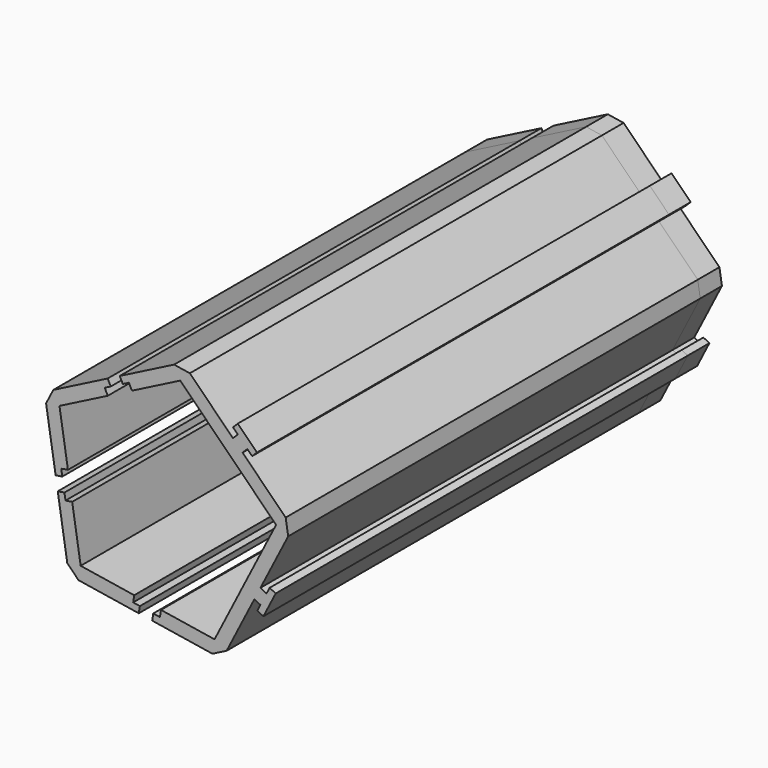
from build123d import *

# Parameters (mm, degrees)
F1_DEPTH = 101.6
F2_DEPTH = 5.08


with BuildPart() as f1:
    # F0 (on Front) → F1 (new body)
    with BuildSketch(Plane.XZ):
        Polygon((-28.6679874819, 40.9869131927), (-27.5148516125, 38.7237566213), (-18.4622253268, 43.3363000986), (-19.0387932615, 44.4678783844), (-17.9072149757, 45.044446319), (-18.4837829104, 46.1760246047), align=None)
        Polygon((-30.0235799977, 38.3264130801), (-27.5148516125, 38.7237566213), (-28.6679874819, 40.9869131927), align=None)
        Polygon((-25.9254774477, 28.6888430808), (-27.5148516125, 38.7237566213), (-30.0235799977, 38.3264130801), (-28.2355340622, 27.0371353471), (-26.9811698697, 27.2358071177), (-27.1798416403, 28.4901713102), align=None)
    extrude(amount=F1_DEPTH)


with BuildPart() as f1b:
    # F0 (on Front) → F1, piece 2 (new body)
    with BuildSketch(Plane.XZ):
        Polygon((-14.5124801186, 46.774150123), (-13.9359121839, 45.6425718373), (-4.8832858982, 50.2551153147), (-6.0364217675, 52.5182718861), (-16.220626339, 47.3291604741), (-15.6440584043, 46.1975821884), align=None)
        Polygon((-6.0364217675, 52.5182718861), (-4.8832858982, 50.2551153147), (-3.0872346739, 52.0511665389), align=None)
        Polygon((-3.0872346739, 52.0511665389), (-4.8832858982, 50.2551153147), (13.077226344, 32.2946030725), (14.8732775682, 34.0906542967), (6.7910470592, 42.1728848057), (7.6890726713, 43.0709104178), (8.5870982834, 42.1728848057), (9.4851238955, 43.0709104178), (5.8930214471, 46.6630128662), (4.994995835, 45.7649872541), (5.8930214471, 44.866961642), (4.994995835, 43.9689360299), align=None)
        Polygon((14.8732775682, 34.0906542967), (13.077226344, 32.2946030725), (15.3403829154, 31.1414672032), align=None)
        Polygon((15.3403829154, 31.1414672032), (13.077226344, 32.2946030725), (1.5458676506, 9.6630373581), (3.809024222, 8.5099014888), (8.9981356341, 18.6941060603), (10.1403821253, 18.138972785), (9.5639359403, 17.0073324729), (10.6955762523, 16.430886288), (13.0017239481, 20.9572626317), (11.8594177238, 21.5122729828), (11.2828497891, 20.3806946971), (10.1512715034, 20.9572626317), align=None)
        Polygon((3.809024222, 8.5099014888), (1.5458676506, 9.6630373581), (1.1485241094, 7.154308973), align=None)
        Polygon((1.5458676506, 9.6630373581), (-8.4890458899, 11.252411523), (-8.6877176605, 9.9980473304), (-9.942081853, 10.196719101), (-10.1407536236, 8.9423549084), (1.1485241094, 7.154308973), align=None)
    extrude(amount=F1_DEPTH)


with BuildPart() as f1c:
    # F0 (on Front) → F1, piece 3 (new body)
    with BuildSketch(Plane.XZ):
        Polygon((-23.9387597417, 11.1277443851), (-23.5414162005, 13.6364727702), (-26.0501445856, 13.239129229), align=None)
        Polygon((-13.5065026601, 12.0470986054), (-23.5414162005, 13.6364727702), (-23.9387597417, 11.1277443851), (-12.6494820087, 9.3396984497), (-12.4508102381, 10.5940626422), (-13.7051744307, 10.7927344128), align=None)
        Polygon((-23.5414162005, 13.6364727702), (-25.1307903653, 23.6713863106), (-26.3851545579, 23.47271454), (-26.5838263285, 24.7270787326), (-27.838190521, 24.528406962), (-26.0501445856, 13.239129229), align=None)
    extrude(amount=F1_DEPTH)


with BuildPart() as f2:
    # F0 (on Front) → F2 (new body)
    with BuildSketch(Plane.XZ):
        Polygon((-18.4622253268, 43.3363000986), (-27.5148516125, 38.7237566213), (-25.9254774477, 28.6888430808), (-25.1307903653, 23.6713863106), (-23.5414162005, 13.6364727702), (-13.5065026601, 12.0470986054), (-8.4890458899, 11.252411523), (1.5458676506, 9.6630373581), (13.077226344, 32.2946030725), (-4.8832858982, 50.2551153147), (-13.9359121839, 45.6425718373), align=None)
        with BuildLine():
            add(Edge.make_bspline(
                [(-24.2410478902, 26.4475166861), (-24.1014147451, 26.5003988632), (-23.9344866256, 26.4169547892)],
                knots=[0, 0, 0, 1, 1, 1], degree=2))
            add(Edge.make_bspline(
                [(-23.9344866256, 26.4169547892), (-23.8245465392, 26.3619979088), (-23.763517385, 26.2778172496)],
                knots=[0, 0, 0, 1, 1, 1], degree=2))
            add(Edge.make_bspline(
                [(-23.763517385, 26.2778172496), (-23.7024882309, 26.1936365905), (-23.6979181512, 26.0929845147)],
                knots=[0, 0, 0, 1, 1, 1], degree=2))
            add(Edge.make_bspline(
                [(-23.6979181512, 26.0929845147), (-23.6933480715, 25.9923324389), (-23.7447541402, 25.8894956767)],
                knots=[0, 0, 0, 1, 1, 1], degree=2))
            Line((-23.7447541402, 25.8894956767), (-23.8776674766, 25.6236053355))
            Line((-23.8776674766, 25.6236053355), (-24.5884842175, 25.9789286021))
            Line((-24.5884842175, 25.9789286021), (-24.4709846317, 26.2139840586))
            add(Edge.make_bspline(
                [(-24.4709846317, 26.2139840586), (-24.3806810352, 26.394634509), (-24.2410478902, 26.4475166861)],
                knots=[0, 0, 0, 1, 1, 1], degree=2))
        make_face(mode=Mode.SUBTRACT)
        with BuildLine():
            Line((-23.5365275255, 26.9405958395), (-23.7311765646, 26.5512045201))
            add(Edge.make_bspline(
                [(-23.7311765646, 26.5512045201), (-23.6373803968, 26.5043176662), (-23.5669572, 26.517642507)],
                knots=[0, 0, 0, 1, 1, 1], degree=2))
            add(Edge.make_bspline(
                [(-23.5669572, 26.517642507), (-23.4965340031, 26.5309673477), (-23.4592504807, 26.6055522522)],
                knots=[0, 0, 0, 1, 1, 1], degree=2))
            add(Edge.make_bspline(
                [(-23.4592504807, 26.6055522522), (-23.4297141837, 26.6646389947), (-23.4356513358, 26.7120992744)],
                knots=[0, 0, 0, 1, 1, 1], degree=2))
            add(Edge.make_bspline(
                [(-23.4356513358, 26.7120992744), (-23.4415884879, 26.7595595541), (-23.4716176843, 26.7903093703)],
                knots=[0, 0, 0, 1, 1, 1], degree=2))
            Line((-23.4716176843, 26.7903093703), (-23.4092309675, 26.8586008524))
            add(Edge.make_bspline(
                [(-23.4092309675, 26.8586008524), (-23.3043703589, 26.7450438665), (-23.3911231438, 26.5714967404)],
                knots=[0, 0, 0, 1, 1, 1], degree=2))
            add(Edge.make_bspline(
                [(-23.3911231438, 26.5714967404), (-23.4516483425, 26.45041735), (-23.555446163, 26.4232062071)],
                knots=[0, 0, 0, 1, 1, 1], degree=2))
            add(Edge.make_bspline(
                [(-23.555446163, 26.4232062071), (-23.6592439835, 26.3959950642), (-23.8016333465, 26.4671726979)],
                knots=[0, 0, 0, 1, 1, 1], degree=2))
            add(Edge.make_bspline(
                [(-23.8016333465, 26.4671726979), (-23.9367579462, 26.5347188197), (-23.9772867589, 26.6340759995)],
                knots=[0, 0, 0, 1, 1, 1], degree=2))
            add(Edge.make_bspline(
                [(-23.9772867589, 26.6340759995), (-24.0178155717, 26.7334331793), (-23.9590657788, 26.8509609075)],
                knots=[0, 0, 0, 1, 1, 1], degree=2))
            add(Edge.make_bspline(
                [(-23.9590657788, 26.8509609075), (-23.8387416837, 27.0916667355), (-23.5486354645, 26.9466483593)],
                knots=[0, 0, 0, 1, 1, 1], degree=2))
            Line((-23.5486354645, 26.9466483593), (-23.5365275255, 26.9405958395))
        make_face(mode=Mode.SUBTRACT)
        with BuildLine():
            add(Edge.make_bspline(
                [(-23.2318323679, 27.4320627384), (-23.2023305644, 27.4299265975), (-23.1710113621, 27.4142707461)],
                knots=[0, 0, 0, 1, 1, 1], degree=2))
            add(Edge.make_bspline(
                [(-23.1710113621, 27.4142707461), (-23.0938434307, 27.3756960194), (-23.0810827573, 27.2964747541)],
                knots=[0, 0, 0, 1, 1, 1], degree=2))
            add(Edge.make_bspline(
                [(-23.0810827573, 27.2964747541), (-23.0683220839, 27.2172534888), (-23.1207772561, 27.1123180172)],
                knots=[0, 0, 0, 1, 1, 1], degree=2))
            add(Edge.make_bspline(
                [(-23.1207772561, 27.1123180172), (-23.1716991233, 27.0104498901), (-23.232918315, 26.9719426237)],
                knots=[0, 0, 0, 1, 1, 1], degree=2))
            add(Edge.make_bspline(
                [(-23.232918315, 26.9719426237), (-23.2941375067, 26.9334353572), (-23.3736443155, 26.9523959378)],
                knots=[0, 0, 0, 1, 1, 1], degree=2))
            Line((-23.3736443155, 26.9523959378), (-23.3491958849, 27.0404591395))
            add(Edge.make_bspline(
                [(-23.3491958849, 27.0404591395), (-23.299474007, 27.0301322889), (-23.2608943902, 27.0562475224)],
                knots=[0, 0, 0, 1, 1, 1], degree=2))
            add(Edge.make_bspline(
                [(-23.2608943902, 27.0562475224), (-23.2223147734, 27.082362756), (-23.1900346674, 27.1469384309)],
                knots=[0, 0, 0, 1, 1, 1], degree=2))
            add(Edge.make_bspline(
                [(-23.1900346674, 27.1469384309), (-23.155494954, 27.216034403), (-23.1606244849, 27.2586518163)],
                knots=[0, 0, 0, 1, 1, 1], degree=2))
            add(Edge.make_bspline(
                [(-23.1606244849, 27.2586518163), (-23.1657540158, 27.3012692297), (-23.208212522, 27.3224933994)],
                knots=[0, 0, 0, 1, 1, 1], degree=2))
            add(Edge.make_bspline(
                [(-23.208212522, 27.3224933994), (-23.2405003595, 27.3386334523), (-23.2717765443, 27.3265230972)],
                knots=[0, 0, 0, 1, 1, 1], degree=2))
            add(Edge.make_bspline(
                [(-23.2717765443, 27.3265230972), (-23.3030527291, 27.3144127421), (-23.3408235843, 27.2715490723)],
                knots=[0, 0, 0, 1, 1, 1], degree=2))
            Line((-23.3408235843, 27.2715490723), (-23.390458345, 27.215043308))
            add(Edge.make_bspline(
                [(-23.390458345, 27.215043308), (-23.4497778719, 27.1468328354), (-23.4857344981, 27.1235429035)],
                knots=[0, 0, 0, 1, 1, 1], degree=2))
            add(Edge.make_bspline(
                [(-23.4857344981, 27.1235429035), (-23.5216911243, 27.1002529717), (-23.5587795451, 27.0954871912)],
                knots=[0, 0, 0, 1, 1, 1], degree=2))
            add(Edge.make_bspline(
                [(-23.5587795451, 27.0954871912), (-23.5958679659, 27.0907214106), (-23.6362277627, 27.1108964769)],
                knots=[0, 0, 0, 1, 1, 1], degree=2))
            add(Edge.make_bspline(
                [(-23.6362277627, 27.1108964769), (-23.7108126671, 27.1481799993), (-23.7232902131, 27.2209036756)],
                knots=[0, 0, 0, 1, 1, 1], degree=2))
            add(Edge.make_bspline(
                [(-23.7232902131, 27.2209036756), (-23.7357677591, 27.2936273518), (-23.6848458919, 27.3954954789)],
                knots=[0, 0, 0, 1, 1, 1], degree=2))
            add(Edge.make_bspline(
                [(-23.6848458919, 27.3954954789), (-23.6396537435, 27.4859014237), (-23.5813402059, 27.5232380338)],
                knots=[0, 0, 0, 1, 1, 1], degree=2))
            add(Edge.make_bspline(
                [(-23.5813402059, 27.5232380338), (-23.5230266683, 27.5605746439), (-23.4457796989, 27.5395152379)],
                knots=[0, 0, 0, 1, 1, 1], degree=2))
            Line((-23.4457796989, 27.5395152379), (-23.4766048034, 27.4528235928))
            add(Edge.make_bspline(
                [(-23.4766048034, 27.4528235928), (-23.5167215329, 27.4633935106), (-23.5525974396, 27.4400632286)],
                knots=[0, 0, 0, 1, 1, 1], degree=2))
            add(Edge.make_bspline(
                [(-23.5525974396, 27.4400632286), (-23.5884733462, 27.4167329467), (-23.6162342374, 27.3611978663)],
                knots=[0, 0, 0, 1, 1, 1], degree=2))
            add(Edge.make_bspline(
                [(-23.6162342374, 27.3611978663), (-23.6469810383, 27.299689536), (-23.6429819103, 27.2610674429)],
                knots=[0, 0, 0, 1, 1, 1], degree=2))
            add(Edge.make_bspline(
                [(-23.6429819103, 27.2610674429), (-23.6389827823, 27.2224453499), (-23.6012060125, 27.2035614879)],
                knots=[0, 0, 0, 1, 1, 1], degree=2))
            add(Edge.make_bspline(
                [(-23.6012060125, 27.2035614879), (-23.5779587695, 27.1919406497), (-23.5568116857, 27.196503114)],
                knots=[0, 0, 0, 1, 1, 1], degree=2))
            add(Edge.make_bspline(
                [(-23.5568116857, 27.196503114), (-23.5356646018, 27.2010655782), (-23.5131466765, 27.2194709213)],
                knots=[0, 0, 0, 1, 1, 1], degree=2))
            add(Edge.make_bspline(
                [(-23.5131466765, 27.2194709213), (-23.4906287512, 27.2378762643), (-23.4339727196, 27.3047950301)],
                knots=[0, 0, 0, 1, 1, 1], degree=2))
            add(Edge.make_bspline(
                [(-23.4339727196, 27.3047950301), (-23.379657073, 27.3678392168), (-23.3484223981, 27.3919762115)],
                knots=[0, 0, 0, 1, 1, 1], degree=2))
            add(Edge.make_bspline(
                [(-23.3484223981, 27.3919762115), (-23.3171877231, 27.4161132062), (-23.2892609472, 27.4251560428)],
                knots=[0, 0, 0, 1, 1, 1], degree=2))
            add(Edge.make_bspline(
                [(-23.2892609472, 27.4251560428), (-23.2613341713, 27.4341988794), (-23.2318323679, 27.4320627384)],
                knots=[0, 0, 0, 1, 1, 1], degree=2))
        make_face(mode=Mode.SUBTRACT)
        Polygon((-22.9216114376, 27.5361753853), (-22.9670456868, 27.4452851229), (-23.5128715784, 27.7181327188), (-23.4674373292, 27.8090229811), align=None, mode=Mode.SUBTRACT)
        Polygon((-23.5835121048, 27.8670464716), (-23.6289463539, 27.7761562093), (-23.7158006366, 27.8195729518), (-23.6703663874, 27.9104632142), align=None, mode=Mode.SUBTRACT)
        with BuildLine():
            add(Edge.make_bspline(
                [(-22.6500587957, 28.1185653779), (-22.4200079541, 28.0035675003), (-22.534198829, 27.7751310506)],
                knots=[0, 0, 0, 1, 1, 1], degree=2))
            add(Edge.make_bspline(
                [(-22.534198829, 27.7751310506), (-22.5789067758, 27.6856937409), (-22.6404087663, 27.650253645)],
                knots=[0, 0, 0, 1, 1, 1], degree=2))
            add(Edge.make_bspline(
                [(-22.6404087663, 27.650253645), (-22.7019107568, 27.6148135492), (-22.7740722566, 27.6319183716)],
                knots=[0, 0, 0, 1, 1, 1], degree=2))
            Line((-22.7740722566, 27.6319183716), (-22.7414724808, 27.7298296729))
            add(Edge.make_bspline(
                [(-22.7414724808, 27.7298296729), (-22.6991764961, 27.7199864054), (-22.663219638, 27.7408548654)],
                knots=[0, 0, 0, 1, 1, 1], degree=2))
            add(Edge.make_bspline(
                [(-22.663219638, 27.7408548654), (-22.6272627798, 27.7617233254), (-22.6020842971, 27.8120923518)],
                knots=[0, 0, 0, 1, 1, 1], degree=2))
            add(Edge.make_bspline(
                [(-22.6020842971, 27.8120923518), (-22.5342153743, 27.9478627082), (-22.6930715344, 28.0272717689)],
                knots=[0, 0, 0, 1, 1, 1], degree=2))
            Line((-22.6930715344, 28.0272717689), (-22.7808944522, 28.071172713))
            Line((-22.7808944522, 28.071172713), (-22.7813786538, 28.0702040779))
            add(Edge.make_bspline(
                [(-22.7813786538, 28.0702040779), (-22.7418229604, 28.0181462218), (-22.7377816073, 27.9600312844)],
                knots=[0, 0, 0, 1, 1, 1], degree=2))
            add(Edge.make_bspline(
                [(-22.7377816073, 27.9600312844), (-22.7337402543, 27.9019163469), (-22.7637607529, 27.8418609693)],
                knots=[0, 0, 0, 1, 1, 1], degree=2))
            add(Edge.make_bspline(
                [(-22.7637607529, 27.8418609693), (-22.8139563177, 27.7414457949), (-22.9041144597, 27.7275944116)],
                knots=[0, 0, 0, 1, 1, 1], degree=2))
            add(Edge.make_bspline(
                [(-22.9041144597, 27.7275944116), (-22.9942726018, 27.7137430282), (-23.1369848432, 27.7850820625)],
                knots=[0, 0, 0, 1, 1, 1], degree=2))
            add(Edge.make_bspline(
                [(-23.1369848432, 27.7850820625), (-23.2817957941, 27.8574702001), (-23.3253097242, 27.9425807679)],
                knots=[0, 0, 0, 1, 1, 1], degree=2))
            add(Edge.make_bspline(
                [(-23.3253097242, 27.9425807679), (-23.3688236543, 28.0276913357), (-23.3170947844, 28.1311738546)],
                knots=[0, 0, 0, 1, 1, 1], degree=2))
            add(Edge.make_bspline(
                [(-23.3170947844, 28.1311738546), (-23.2881233893, 28.1891305228), (-23.2403424927, 28.2185156247)],
                knots=[0, 0, 0, 1, 1, 1], degree=2))
            add(Edge.make_bspline(
                [(-23.2403424927, 28.2185156247), (-23.192561596, 28.2479007267), (-23.1320246842, 28.2466957893)],
                knots=[0, 0, 0, 1, 1, 1], degree=2))
            Line((-23.1320246842, 28.2466957893), (-23.1315404826, 28.2476644244))
            add(Edge.make_bspline(
                [(-23.1315404826, 28.2476644244), (-23.1467157662, 28.2552502494), (-23.1829994651, 28.2759100004)],
                knots=[0, 0, 0, 1, 1, 1], degree=2))
            add(Edge.make_bspline(
                [(-23.1829994651, 28.2759100004), (-23.219283164, 28.2965697514), (-23.2217857227, 28.3004438667)],
                knots=[0, 0, 0, 1, 1, 1], degree=2))
            Line((-23.2217857227, 28.3004438667), (-23.1786917812, 28.3866523926))
            add(Edge.make_bspline(
                [(-23.1786917812, 28.3866523926), (-23.1531033028, 28.3700274036), (-23.0672176552, 28.3270948626)],
                knots=[0, 0, 0, 1, 1, 1], degree=2))
            Line((-23.0672176552, 28.3270948626), (-22.6500587957, 28.1185653779))
        make_face(mode=Mode.SUBTRACT)
        with BuildLine():
            Line((-22.3458957473, 28.6878825462), (-22.3915720973, 28.5965079663))
            Line((-22.3915720973, 28.5965079663), (-22.7376977145, 28.7695293343))
            add(Edge.make_bspline(
                [(-22.7376977145, 28.7695293343), (-22.791618403, 28.7964832228), (-22.8266898003, 28.800798155)],
                knots=[0, 0, 0, 1, 1, 1], degree=2))
            add(Edge.make_bspline(
                [(-22.8266898003, 28.800798155), (-22.8617611977, 28.8051130871), (-22.88645861, 28.7884025656)],
                knots=[0, 0, 0, 1, 1, 1], degree=2))
            add(Edge.make_bspline(
                [(-22.88645861, 28.7884025656), (-22.9111560223, 28.7716920441), (-22.933590696, 28.7268119501)],
                knots=[0, 0, 0, 1, 1, 1], degree=2))
            add(Edge.make_bspline(
                [(-22.933590696, 28.7268119501), (-22.9663550036, 28.6612676402), (-22.9403991217, 28.6009754771)],
                knots=[0, 0, 0, 1, 1, 1], degree=2))
            add(Edge.make_bspline(
                [(-22.9403991217, 28.6009754771), (-22.9144432398, 28.5406833141), (-22.8346922814, 28.5008173832)],
                knots=[0, 0, 0, 1, 1, 1], degree=2))
            Line((-22.8346922814, 28.5008173832), (-22.5184329138, 28.3427255641))
            Line((-22.5184329138, 28.3427255641), (-22.5637864627, 28.251996741))
            Line((-22.5637864627, 28.251996741), (-22.9930532613, 28.4665787455))
            add(Edge.make_bspline(
                [(-22.9930532613, 28.4665787455), (-23.0884638209, 28.5142726021), (-23.1111456594, 28.5217769922)],
                knots=[0, 0, 0, 1, 1, 1], degree=2))
            Line((-23.1111456594, 28.5217769922), (-23.0682938187, 28.6075012006))
            add(Edge.make_bspline(
                [(-23.0682938187, 28.6075012006), (-23.0656301301, 28.6067750142), (-23.0542083753, 28.6017717331)],
                knots=[0, 0, 0, 1, 1, 1], degree=2))
            add(Edge.make_bspline(
                [(-23.0542083753, 28.6017717331), (-23.0427866204, 28.5967684519), (-23.0280553816, 28.5903126047)],
                knots=[0, 0, 0, 1, 1, 1], degree=2))
            add(Edge.make_bspline(
                [(-23.0280553816, 28.5903126047), (-23.0133241427, 28.5838567575), (-22.9729644619, 28.5648924271)],
                knots=[0, 0, 0, 1, 1, 1], degree=2))
            Line((-22.9729644619, 28.5648924271), (-22.9721574593, 28.566506819))
            add(Edge.make_bspline(
                [(-22.9721574593, 28.566506819), (-23.0130860236, 28.6259096749), (-23.0159968578, 28.6788185561)],
                knots=[0, 0, 0, 1, 1, 1], degree=2))
            add(Edge.make_bspline(
                [(-23.0159968578, 28.6788185561), (-23.0189076919, 28.7317274374), (-22.9884029918, 28.7927514501)],
                knots=[0, 0, 0, 1, 1, 1], degree=2))
            add(Edge.make_bspline(
                [(-22.9884029918, 28.7927514501), (-22.9435336445, 28.8825116382), (-22.8780750409, 28.9018493252)],
                knots=[0, 0, 0, 1, 1, 1], degree=2))
            add(Edge.make_bspline(
                [(-22.8780750409, 28.9018493252), (-22.8126164373, 28.9211870122), (-22.7096182359, 28.8697002431)],
                knots=[0, 0, 0, 1, 1, 1], degree=2))
            Line((-22.7096182359, 28.8697002431), (-22.3458957473, 28.6878825462))
        make_face(mode=Mode.SUBTRACT)
        with BuildLine():
            Line((-22.3018941717, 29.4104539632), (-22.4965432108, 29.0210626438))
            add(Edge.make_bspline(
                [(-22.4965432108, 29.0210626438), (-22.4027470431, 28.9741757899), (-22.3323238463, 28.9875006307)],
                knots=[0, 0, 0, 1, 1, 1], degree=2))
            add(Edge.make_bspline(
                [(-22.3323238463, 28.9875006307), (-22.2619006494, 29.0008254714), (-22.224617127, 29.0754103759)],
                knots=[0, 0, 0, 1, 1, 1], degree=2))
            add(Edge.make_bspline(
                [(-22.224617127, 29.0754103759), (-22.19508083, 29.1344971184), (-22.2010179821, 29.1819573981)],
                knots=[0, 0, 0, 1, 1, 1], degree=2))
            add(Edge.make_bspline(
                [(-22.2010179821, 29.1819573981), (-22.2069551342, 29.2294176778), (-22.2369843306, 29.260167494)],
                knots=[0, 0, 0, 1, 1, 1], degree=2))
            Line((-22.2369843306, 29.260167494), (-22.1745976138, 29.3284589761))
            add(Edge.make_bspline(
                [(-22.1745976138, 29.3284589761), (-22.0697370052, 29.2149019902), (-22.15648979, 29.0413548641)],
                knots=[0, 0, 0, 1, 1, 1], degree=2))
            add(Edge.make_bspline(
                [(-22.15648979, 29.0413548641), (-22.2170149888, 28.9202754737), (-22.3208128093, 28.8930643308)],
                knots=[0, 0, 0, 1, 1, 1], degree=2))
            add(Edge.make_bspline(
                [(-22.3208128093, 28.8930643308), (-22.4246106298, 28.8658531879), (-22.5669999928, 28.9370308216)],
                knots=[0, 0, 0, 1, 1, 1], degree=2))
            add(Edge.make_bspline(
                [(-22.5669999928, 28.9370308216), (-22.7021245924, 29.0045769434), (-22.7426534052, 29.1039341232)],
                knots=[0, 0, 0, 1, 1, 1], degree=2))
            add(Edge.make_bspline(
                [(-22.7426534052, 29.1039341232), (-22.783182218, 29.203291303), (-22.7244324251, 29.3208190312)],
                knots=[0, 0, 0, 1, 1, 1], degree=2))
            add(Edge.make_bspline(
                [(-22.7244324251, 29.3208190312), (-22.60410833, 29.5615248592), (-22.3140021108, 29.416506483)],
                knots=[0, 0, 0, 1, 1, 1], degree=2))
            Line((-22.3140021108, 29.416506483), (-22.3018941717, 29.4104539632))
        make_face(mode=Mode.SUBTRACT)
        with BuildLine():
            Line((-21.9049705291, 29.7895330443), (-21.9059389322, 29.7875957741))
            add(Edge.make_bspline(
                [(-21.9059389322, 29.7875957741), (-21.866141138, 29.7360222356), (-21.8641585309, 29.6830729075)],
                knots=[0, 0, 0, 1, 1, 1], degree=2))
            add(Edge.make_bspline(
                [(-21.8641585309, 29.6830729075), (-21.8621759237, 29.6301235795), (-21.8929227247, 29.5686152492)],
                knots=[0, 0, 0, 1, 1, 1], degree=2))
            add(Edge.make_bspline(
                [(-21.8929227247, 29.5686152492), (-21.9446515945, 29.4651327302), (-22.0386437336, 29.4512809797)],
                knots=[0, 0, 0, 1, 1, 1], degree=2))
            add(Edge.make_bspline(
                [(-22.0386437336, 29.4512809797), (-22.1326358728, 29.4374292291), (-22.2738951615, 29.5080419609)],
                knots=[0, 0, 0, 1, 1, 1], degree=2))
            add(Edge.make_bspline(
                [(-22.2738951615, 29.5080419609), (-22.5594810835, 29.6508007296), (-22.4590899539, 29.8516310784)],
                knots=[0, 0, 0, 1, 1, 1], degree=2))
            add(Edge.make_bspline(
                [(-22.4590899539, 29.8516310784), (-22.4281010521, 29.9136237263), (-22.3847595785, 29.9436137709)],
                knots=[0, 0, 0, 1, 1, 1], degree=2))
            add(Edge.make_bspline(
                [(-22.3847595785, 29.9436137709), (-22.3414181049, 29.9736038156), (-22.2791863328, 29.9741747867)],
                knots=[0, 0, 0, 1, 1, 1], degree=2))
            Line((-22.2791863328, 29.9741747867), (-22.2787021313, 29.9751434218))
            Line((-22.2787021313, 29.9751434218), (-22.3402103456, 30.0046794868))
            Line((-22.3402103456, 30.0046794868), (-22.5668709643, 30.1179826588))
            Line((-22.5668709643, 30.1179826588), (-22.5215174154, 30.208711482))
            Line((-22.5215174154, 30.208711482), (-21.8852855789, 29.8906717378))
            add(Edge.make_bspline(
                [(-21.8852855789, 29.8906717378), (-21.8000456882, 29.8480619979), (-21.7712291605, 29.8374909976)],
                knots=[0, 0, 0, 1, 1, 1], degree=2))
            Line((-21.7712291605, 29.8374909976), (-21.814645903, 29.750636715))
            add(Edge.make_bspline(
                [(-21.814645903, 29.750636715), (-21.8234441648, 29.7532187755), (-21.8536330802, 29.7660900426)],
                knots=[0, 0, 0, 1, 1, 1], degree=2))
            add(Edge.make_bspline(
                [(-21.8536330802, 29.7660900426), (-21.8838219955, 29.7789613096), (-21.9049705291, 29.7895330443)],
                knots=[0, 0, 0, 1, 1, 1], degree=2))
        make_face(mode=Mode.SUBTRACT)
        with BuildLine():
            add(Edge.make_bspline(
                [(-21.8395776893, 30.9167748155), (-21.7455855502, 30.9306265661), (-21.6043262614, 30.8600138342)],
                knots=[0, 0, 0, 1, 1, 1], degree=2))
            add(Edge.make_bspline(
                [(-21.6043262614, 30.8600138342), (-21.3187403394, 30.7172550655), (-21.419131469, 30.5164247168)],
                knots=[0, 0, 0, 1, 1, 1], degree=2))
            add(Edge.make_bspline(
                [(-21.419131469, 30.5164247168), (-21.4501203708, 30.4544320689), (-21.493219705, 30.4245227631)],
                knots=[0, 0, 0, 1, 1, 1], degree=2))
            add(Edge.make_bspline(
                [(-21.493219705, 30.4245227631), (-21.5363190391, 30.3946134574), (-21.5990350901, 30.3938810085)],
                knots=[0, 0, 0, 1, 1, 1], degree=2))
            Line((-21.5990350901, 30.3938810085), (-21.5995192917, 30.3929123734))
            add(Edge.make_bspline(
                [(-21.5995192917, 30.3929123734), (-21.5838596905, 30.3850844477), (-21.5528227652, 30.3670474553)],
                knots=[0, 0, 0, 1, 1, 1], degree=2))
            add(Edge.make_bspline(
                [(-21.5528227652, 30.3670474553), (-21.5217858399, 30.3490104628), (-21.5173461269, 30.3453786803)],
                knots=[0, 0, 0, 1, 1, 1], degree=2))
            Line((-21.5173461269, 30.3453786803), (-21.5611663708, 30.2577172017))
            add(Edge.make_bspline(
                [(-21.5611663708, 30.2577172017), (-21.5869969886, 30.2742614518), (-21.6722368794, 30.3168711917)],
                knots=[0, 0, 0, 1, 1, 1], degree=2))
            Line((-21.6722368794, 30.3168711917), (-22.3084687159, 30.634910936))
            Line((-22.3084687159, 30.634910936), (-22.2630344667, 30.7258011983))
            Line((-22.2630344667, 30.7258011983), (-22.0496118613, 30.619115448))
            add(Edge.make_bspline(
                [(-22.0496118613, 30.619115448), (-22.0168397063, 30.6027332942), (-21.9734930333, 30.578442012)],
                knots=[0, 0, 0, 1, 1, 1], degree=2))
            Line((-21.9734930333, 30.578442012), (-21.9724439299, 30.5805407214))
            add(Edge.make_bspline(
                [(-21.9724439299, 30.5805407214), (-22.0123224244, 30.6319528207), (-22.0141839618, 30.6849425182)],
                knots=[0, 0, 0, 1, 1, 1], degree=2))
            add(Edge.make_bspline(
                [(-22.0141839618, 30.6849425182), (-22.0160454992, 30.7379322157), (-21.9852986983, 30.799440546)],
                knots=[0, 0, 0, 1, 1, 1], degree=2))
            add(Edge.make_bspline(
                [(-21.9852986983, 30.799440546), (-21.9335698284, 30.9029230649), (-21.8395776893, 30.9167748155)],
                knots=[0, 0, 0, 1, 1, 1], degree=2))
        make_face(mode=Mode.SUBTRACT)
        with BuildLine():
            add(Edge.make_bspline(
                [(-21.0253913312, 30.8457422463), (-21.0222793649, 30.7996942212), (-21.0447140385, 30.7548141272)],
                knots=[0, 0, 0, 1, 1, 1], degree=2))
            add(Edge.make_bspline(
                [(-21.0447140385, 30.7548141272), (-21.0633557997, 30.717521675), (-21.0815146737, 30.6949195316)],
                knots=[0, 0, 0, 1, 1, 1], degree=2))
            Line((-21.0815146737, 30.6949195316), (-21.1496420107, 30.7289750434))
            add(Edge.make_bspline(
                [(-21.1496420107, 30.7289750434), (-21.1369713346, 30.7466530017), (-21.1253504964, 30.7699002446)],
                knots=[0, 0, 0, 1, 1, 1], degree=2))
            add(Edge.make_bspline(
                [(-21.1253504964, 30.7699002446), (-21.0829828573, 30.8546558178), (-21.1829196287, 30.9663568136)],
                knots=[0, 0, 0, 1, 1, 1], degree=2))
            Line((-21.1829196287, 30.9663568136), (-21.2004368049, 30.9858076263))
            Line((-21.2004368049, 30.9858076263), (-21.8518180246, 31.0410355072))
            Line((-21.8518180246, 31.0410355072), (-21.8033978656, 31.1378990195))
            Line((-21.8033978656, 31.1378990195), (-21.4443708754, 31.1020956257))
            add(Edge.make_bspline(
                [(-21.4443708754, 31.1020956257), (-21.435976347, 31.1011278411), (-21.4243531507, 31.099756787)],
                knots=[0, 0, 0, 1, 1, 1], degree=2))
            add(Edge.make_bspline(
                [(-21.4243531507, 31.099756787), (-21.4127299545, 31.098385733), (-21.3471475751, 31.0895132847)],
                knots=[0, 0, 0, 1, 1, 1], degree=2))
            add(Edge.make_bspline(
                [(-21.3471475751, 31.0895132847), (-21.2815651958, 31.0806408365), (-21.274381326, 31.0788657785)],
                knots=[0, 0, 0, 1, 1, 1], degree=2))
            Line((-21.274381326, 31.0788657785), (-21.355993068, 31.1638516235))
            Line((-21.355993068, 31.1638516235), (-21.6437727415, 31.4572257316))
            Line((-21.6437727415, 31.4572257316), (-21.5958367841, 31.5531206087))
            Line((-21.5958367841, 31.5531206087), (-21.1549212369, 31.0704020696))
            add(Edge.make_bspline(
                [(-21.1549212369, 31.0704020696), (-21.0845296924, 30.992840997), (-21.0565164949, 30.9423156342)],
                knots=[0, 0, 0, 1, 1, 1], degree=2))
            add(Edge.make_bspline(
                [(-21.0565164949, 30.9423156342), (-21.0285032975, 30.8917902714), (-21.0253913312, 30.8457422463)],
                knots=[0, 0, 0, 1, 1, 1], degree=2))
        make_face(mode=Mode.SUBTRACT)
        with BuildLine():
            add(Edge.make_bspline(
                [(-20.7628104206, 31.9777247755), (-20.7314845113, 31.8920480302), (-20.780146771, 31.7947002003)],
                knots=[0, 0, 0, 1, 1, 1], degree=2))
            add(Edge.make_bspline(
                [(-20.780146771, 31.7947002003), (-20.8704503675, 31.61404975), (-21.0741018624, 31.6736791664)],
                knots=[0, 0, 0, 1, 1, 1], degree=2))
            Line((-21.0741018624, 31.6736791664), (-21.0426325088, 31.7757875774))
            add(Edge.make_bspline(
                [(-21.0426325088, 31.7757875774), (-20.9794301688, 31.7556954149), (-20.9308004117, 31.7710360614)],
                knots=[0, 0, 0, 1, 1, 1], degree=2))
            add(Edge.make_bspline(
                [(-20.9308004117, 31.7710360614), (-20.8821706547, 31.7863767078), (-20.858202676, 31.8343241464)],
                knots=[0, 0, 0, 1, 1, 1], degree=2))
            add(Edge.make_bspline(
                [(-20.858202676, 31.8343241464), (-20.8319750899, 31.8867918822), (-20.8529254485, 31.935098239)],
                knots=[0, 0, 0, 1, 1, 1], degree=2))
            add(Edge.make_bspline(
                [(-20.8529254485, 31.935098239), (-20.8738758072, 31.9834045958), (-20.9434560968, 32.01818641)],
                knots=[0, 0, 0, 1, 1, 1], degree=2))
            Line((-20.9434560968, 32.01818641), (-21.3657810103, 32.2292983032))
            Line((-21.3657810103, 32.2292983032), (-21.4341341347, 32.0925593117))
            Line((-21.4341341347, 32.0925593117), (-21.5127550189, 32.1318603407))
            Line((-21.5127550189, 32.1318603407), (-21.396465937, 32.3644942094))
            Line((-21.396465937, 32.3644942094), (-20.8976188489, 32.1151303906))
            add(Edge.make_bspline(
                [(-20.8976188489, 32.1151303906), (-20.7941363299, 32.0634015208), (-20.7628104206, 31.9777247755)],
                knots=[0, 0, 0, 1, 1, 1], degree=2))
        make_face(mode=Mode.SUBTRACT)
        with BuildLine():
            Line((-20.6368056047, 32.7414287109), (-20.8314546438, 32.3520373916))
            add(Edge.make_bspline(
                [(-20.8314546438, 32.3520373916), (-20.7376584761, 32.3051505377), (-20.6672352792, 32.3184753784)],
                knots=[0, 0, 0, 1, 1, 1], degree=2))
            add(Edge.make_bspline(
                [(-20.6672352792, 32.3184753784), (-20.5968120824, 32.3318002192), (-20.55952856, 32.4063851237)],
                knots=[0, 0, 0, 1, 1, 1], degree=2))
            add(Edge.make_bspline(
                [(-20.55952856, 32.4063851237), (-20.529992263, 32.4654718661), (-20.5359294151, 32.5129321459)],
                knots=[0, 0, 0, 1, 1, 1], degree=2))
            add(Edge.make_bspline(
                [(-20.5359294151, 32.5129321459), (-20.5418665671, 32.5603924256), (-20.5718957636, 32.5911422418)],
                knots=[0, 0, 0, 1, 1, 1], degree=2))
            Line((-20.5718957636, 32.5911422418), (-20.5095090467, 32.6594337239))
            add(Edge.make_bspline(
                [(-20.5095090467, 32.6594337239), (-20.4046484382, 32.545876738), (-20.491401223, 32.3723296118)],
                knots=[0, 0, 0, 1, 1, 1], degree=2))
            add(Edge.make_bspline(
                [(-20.491401223, 32.3723296118), (-20.5519264217, 32.2512502215), (-20.6557242422, 32.2240390786)],
                knots=[0, 0, 0, 1, 1, 1], degree=2))
            add(Edge.make_bspline(
                [(-20.6557242422, 32.2240390786), (-20.7595220627, 32.1968279357), (-20.9019114258, 32.2680055694)],
                knots=[0, 0, 0, 1, 1, 1], degree=2))
            add(Edge.make_bspline(
                [(-20.9019114258, 32.2680055694), (-21.0370360254, 32.3355516912), (-21.0775648382, 32.434908871)],
                knots=[0, 0, 0, 1, 1, 1], degree=2))
            add(Edge.make_bspline(
                [(-21.0775648382, 32.434908871), (-21.1180936509, 32.5342660507), (-21.059343858, 32.651793779)],
                knots=[0, 0, 0, 1, 1, 1], degree=2))
            add(Edge.make_bspline(
                [(-21.059343858, 32.651793779), (-20.939019763, 32.892499607), (-20.6489135437, 32.7474812308)],
                knots=[0, 0, 0, 1, 1, 1], degree=2))
            Line((-20.6489135437, 32.7474812308), (-20.6368056047, 32.7414287109))
        make_face(mode=Mode.SUBTRACT)
        with BuildLine():
            Line((-20.6956095176, 33.1889110776), (-20.7488716925, 33.0823612141))
            Line((-20.7488716925, 33.0823612141), (-20.2690744284, 32.8425200266))
            Line((-20.2690744284, 32.8425200266), (-20.3144279773, 32.7517912035))
            Line((-20.3144279773, 32.7517912035), (-20.7942252414, 32.9916323909))
            Line((-20.7942252414, 32.9916323909), (-20.8325578673, 32.9149487771))
            Line((-20.8325578673, 32.9149487771), (-20.8985864948, 32.9479551854))
            Line((-20.8985864948, 32.9479551854), (-20.860253869, 33.0246387993))
            Line((-20.860253869, 33.0246387993), (-20.9219236384, 33.0554663005))
            add(Edge.make_bspline(
                [(-20.9219236384, 33.0554663005), (-20.9965085429, 33.0927498229), (-21.0128985441, 33.1419041317)],
                knots=[0, 0, 0, 1, 1, 1], degree=2))
            add(Edge.make_bspline(
                [(-21.0128985441, 33.1419041317), (-21.0292885453, 33.1910584405), (-20.9954751343, 33.2587014599)],
                knots=[0, 0, 0, 1, 1, 1], degree=2))
            add(Edge.make_bspline(
                [(-20.9954751343, 33.2587014599), (-20.9765912723, 33.2964782297), (-20.9574638791, 33.3198069074)],
                knots=[0, 0, 0, 1, 1, 1], degree=2))
            Line((-20.9574638791, 33.3198069074), (-20.8883679071, 33.285267194))
            add(Edge.make_bspline(
                [(-20.8883679071, 33.285267194), (-20.9037826241, 33.2645217752), (-20.912578953, 33.2469249038)],
                knots=[0, 0, 0, 1, 1, 1], degree=2))
            add(Edge.make_bspline(
                [(-20.912578953, 33.2469249038), (-20.9300102102, 33.2120540394), (-20.9201605449, 33.1875577592)],
                knots=[0, 0, 0, 1, 1, 1], degree=2))
            add(Edge.make_bspline(
                [(-20.9201605449, 33.1875577592), (-20.9103108796, 33.1630614791), (-20.8638163938, 33.1398198028)],
                knots=[0, 0, 0, 1, 1, 1], degree=2))
            Line((-20.8638163938, 33.1398198028), (-20.8149003201, 33.1153676225))
            Line((-20.8149003201, 33.1153676225), (-20.7616381452, 33.221917486))
            Line((-20.7616381452, 33.221917486), (-20.6956095176, 33.1889110776))
        make_face(mode=Mode.SUBTRACT)
        with BuildLine():
            Line((-20.5521244465, 33.4759499523), (-20.6053866214, 33.3694000888))
            Line((-20.6053866214, 33.3694000888), (-20.1255893573, 33.1295589013))
            Line((-20.1255893573, 33.1295589013), (-20.1709429062, 33.0388300782))
            Line((-20.1709429062, 33.0388300782), (-20.6507401703, 33.2786712656))
            Line((-20.6507401703, 33.2786712656), (-20.6890727962, 33.2019876518))
            Line((-20.6890727962, 33.2019876518), (-20.7551014237, 33.2349940601))
            Line((-20.7551014237, 33.2349940601), (-20.7167687979, 33.311677674))
            Line((-20.7167687979, 33.311677674), (-20.7784385673, 33.3425051752))
            add(Edge.make_bspline(
                [(-20.7784385673, 33.3425051752), (-20.8530234718, 33.3797886976), (-20.869413473, 33.4289430064)],
                knots=[0, 0, 0, 1, 1, 1], degree=2))
            add(Edge.make_bspline(
                [(-20.869413473, 33.4289430064), (-20.8858034742, 33.4780973152), (-20.8519900632, 33.5457403346)],
                knots=[0, 0, 0, 1, 1, 1], degree=2))
            add(Edge.make_bspline(
                [(-20.8519900632, 33.5457403346), (-20.8331062012, 33.5835171044), (-20.813978808, 33.6068457821)],
                knots=[0, 0, 0, 1, 1, 1], degree=2))
            Line((-20.813978808, 33.6068457821), (-20.744882836, 33.5723060687))
            add(Edge.make_bspline(
                [(-20.744882836, 33.5723060687), (-20.760297553, 33.5515606499), (-20.7690938819, 33.5339637785)],
                knots=[0, 0, 0, 1, 1, 1], degree=2))
            add(Edge.make_bspline(
                [(-20.7690938819, 33.5339637785), (-20.7865251391, 33.4990929141), (-20.7766754738, 33.4745966339)],
                knots=[0, 0, 0, 1, 1, 1], degree=2))
            add(Edge.make_bspline(
                [(-20.7766754738, 33.4745966339), (-20.7668258085, 33.4501003538), (-20.7203313226, 33.4268586775)],
                knots=[0, 0, 0, 1, 1, 1], degree=2))
            Line((-20.7203313226, 33.4268586775), (-20.6714152489, 33.4024064972))
            Line((-20.6714152489, 33.4024064972), (-20.6181530741, 33.5089563607))
            Line((-20.6181530741, 33.5089563607), (-20.5521244465, 33.4759499523))
        make_face(mode=Mode.SUBTRACT)
        with BuildLine():
            Line((-20.0626232195, 33.8900685273), (-20.2572722586, 33.500677208))
            add(Edge.make_bspline(
                [(-20.2572722586, 33.500677208), (-20.1634760908, 33.453790354), (-20.093052894, 33.4671151948)],
                knots=[0, 0, 0, 1, 1, 1], degree=2))
            add(Edge.make_bspline(
                [(-20.093052894, 33.4671151948), (-20.0226296971, 33.4804400356), (-19.9853461747, 33.55502494)],
                knots=[0, 0, 0, 1, 1, 1], degree=2))
            add(Edge.make_bspline(
                [(-19.9853461747, 33.55502494), (-19.9558098777, 33.6141116825), (-19.9617470298, 33.6615719622)],
                knots=[0, 0, 0, 1, 1, 1], degree=2))
            add(Edge.make_bspline(
                [(-19.9617470298, 33.6615719622), (-19.9676841819, 33.7090322419), (-19.9977133783, 33.7397820581)],
                knots=[0, 0, 0, 1, 1, 1], degree=2))
            Line((-19.9977133783, 33.7397820581), (-19.9353266615, 33.8080735403))
            add(Edge.make_bspline(
                [(-19.9353266615, 33.8080735403), (-19.8304660529, 33.6945165543), (-19.9172188378, 33.5209694282)],
                knots=[0, 0, 0, 1, 1, 1], degree=2))
            add(Edge.make_bspline(
                [(-19.9172188378, 33.5209694282), (-19.9777440365, 33.3998900378), (-20.081541857, 33.3726788949)],
                knots=[0, 0, 0, 1, 1, 1], degree=2))
            add(Edge.make_bspline(
                [(-20.081541857, 33.3726788949), (-20.1853396775, 33.345467752), (-20.3277290405, 33.4166453857)],
                knots=[0, 0, 0, 1, 1, 1], degree=2))
            add(Edge.make_bspline(
                [(-20.3277290405, 33.4166453857), (-20.4628536402, 33.4841915075), (-20.5033824529, 33.5835486873)],
                knots=[0, 0, 0, 1, 1, 1], degree=2))
            add(Edge.make_bspline(
                [(-20.5033824529, 33.5835486873), (-20.5439112657, 33.6829058671), (-20.4851614728, 33.8004335953)],
                knots=[0, 0, 0, 1, 1, 1], degree=2))
            add(Edge.make_bspline(
                [(-20.4851614728, 33.8004335953), (-20.3648373777, 34.0411394233), (-20.0747311585, 33.8961210472)],
                knots=[0, 0, 0, 1, 1, 1], degree=2))
            Line((-20.0747311585, 33.8961210472), (-20.0626232195, 33.8900685273))
        make_face(mode=Mode.SUBTRACT)
        with BuildLine():
            Line((-19.7047374755, 33.9714642621), (-19.7500910244, 33.880735439))
            Line((-19.7500910244, 33.880735439), (-20.1688642758, 34.0900719263))
            add(Edge.make_bspline(
                [(-20.1688642758, 34.0900719263), (-20.2263366264, 34.1188012206), (-20.2974502211, 34.1505156903)],
                knots=[0, 0, 0, 1, 1, 1], degree=2))
            Line((-20.2974502211, 34.1505156903), (-20.2545983804, 34.2362398986))
            add(Edge.make_bspline(
                [(-20.2545983804, 34.2362398986), (-20.1597533412, 34.193873226), (-20.1411878347, 34.1845926955)],
                knots=[0, 0, 0, 1, 1, 1], degree=2))
            Line((-20.1411878347, 34.1845926955), (-20.1401387312, 34.1866914049))
            add(Edge.make_bspline(
                [(-20.1401387312, 34.1866914049), (-20.1993895029, 34.243348171), (-20.2110165069, 34.284471721)],
                knots=[0, 0, 0, 1, 1, 1], degree=2))
            add(Edge.make_bspline(
                [(-20.2110165069, 34.284471721), (-20.2226435109, 34.325595271), (-20.1969001263, 34.3770943717)],
                knots=[0, 0, 0, 1, 1, 1], degree=2))
            add(Edge.make_bspline(
                [(-20.1969001263, 34.3770943717), (-20.1878616967, 34.3951755606), (-20.1734958511, 34.4114007981)],
                knots=[0, 0, 0, 1, 1, 1], degree=2))
            Line((-20.1734958511, 34.4114007981), (-20.0901932306, 34.3697594614))
            add(Edge.make_bspline(
                [(-20.0901932306, 34.3697594614), (-20.1042362751, 34.3541799807), (-20.1194079249, 34.3238294135)],
                knots=[0, 0, 0, 1, 1, 1], degree=2))
            add(Edge.make_bspline(
                [(-20.1194079249, 34.3238294135), (-20.1476530176, 34.267325698), (-20.1138683016, 34.2132090381)],
                knots=[0, 0, 0, 1, 1, 1], degree=2))
            add(Edge.make_bspline(
                [(-20.1138683016, 34.2132090381), (-20.0800835856, 34.1590923782), (-19.9893547624, 34.1137388293)],
                knots=[0, 0, 0, 1, 1, 1], degree=2))
            Line((-19.9893547624, 34.1137388293), (-19.7047374755, 33.9714642621))
        make_face(mode=Mode.SUBTRACT)
        with BuildLine():
            add(Edge.make_bspline(
                [(-19.5859557972, 34.725562334), (-19.5564539938, 34.7234261931), (-19.5251347915, 34.7077703417)],
                knots=[0, 0, 0, 1, 1, 1], degree=2))
            add(Edge.make_bspline(
                [(-19.5251347915, 34.7077703417), (-19.4479668601, 34.669195615), (-19.4352061867, 34.5899743497)],
                knots=[0, 0, 0, 1, 1, 1], degree=2))
            add(Edge.make_bspline(
                [(-19.4352061867, 34.5899743497), (-19.4224455132, 34.5107530844), (-19.4749006855, 34.4058176128)],
                knots=[0, 0, 0, 1, 1, 1], degree=2))
            add(Edge.make_bspline(
                [(-19.4749006855, 34.4058176128), (-19.5258225527, 34.3039494857), (-19.5870417443, 34.2654422192)],
                knots=[0, 0, 0, 1, 1, 1], degree=2))
            add(Edge.make_bspline(
                [(-19.5870417443, 34.2654422192), (-19.648260936, 34.2269349528), (-19.7277677448, 34.2458955333)],
                knots=[0, 0, 0, 1, 1, 1], degree=2))
            Line((-19.7277677448, 34.2458955333), (-19.7033193143, 34.333958735))
            add(Edge.make_bspline(
                [(-19.7033193143, 34.333958735), (-19.6535974363, 34.3236318844), (-19.6150178195, 34.349747118)],
                knots=[0, 0, 0, 1, 1, 1], degree=2))
            add(Edge.make_bspline(
                [(-19.6150178195, 34.349747118), (-19.5764382027, 34.3758623516), (-19.5441580967, 34.4404380264)],
                knots=[0, 0, 0, 1, 1, 1], degree=2))
            add(Edge.make_bspline(
                [(-19.5441580967, 34.4404380264), (-19.5096183833, 34.5095339985), (-19.5147479143, 34.5521514119)],
                knots=[0, 0, 0, 1, 1, 1], degree=2))
            add(Edge.make_bspline(
                [(-19.5147479143, 34.5521514119), (-19.5198774452, 34.5947688252), (-19.5623359514, 34.6159929949)],
                knots=[0, 0, 0, 1, 1, 1], degree=2))
            add(Edge.make_bspline(
                [(-19.5623359514, 34.6159929949), (-19.5946237888, 34.6321330479), (-19.6258999736, 34.6200226928)],
                knots=[0, 0, 0, 1, 1, 1], degree=2))
            add(Edge.make_bspline(
                [(-19.6258999736, 34.6200226928), (-19.6571761585, 34.6079123377), (-19.6949470137, 34.5650486679)],
                knots=[0, 0, 0, 1, 1, 1], degree=2))
            Line((-19.6949470137, 34.5650486679), (-19.7445817743, 34.5085429036))
            add(Edge.make_bspline(
                [(-19.7445817743, 34.5085429036), (-19.8039013012, 34.440332431), (-19.8398579274, 34.4170424991)],
                knots=[0, 0, 0, 1, 1, 1], degree=2))
            add(Edge.make_bspline(
                [(-19.8398579274, 34.4170424991), (-19.8758145537, 34.3937525673), (-19.9129029745, 34.3889867867)],
                knots=[0, 0, 0, 1, 1, 1], degree=2))
            add(Edge.make_bspline(
                [(-19.9129029745, 34.3889867867), (-19.9499913952, 34.3842210062), (-19.990351192, 34.4043960724)],
                knots=[0, 0, 0, 1, 1, 1], degree=2))
            add(Edge.make_bspline(
                [(-19.990351192, 34.4043960724), (-20.0649360965, 34.4416795949), (-20.0774136425, 34.5144032711)],
                knots=[0, 0, 0, 1, 1, 1], degree=2))
            add(Edge.make_bspline(
                [(-20.0774136425, 34.5144032711), (-20.0898911884, 34.5871269474), (-20.0389693212, 34.6889950745)],
                knots=[0, 0, 0, 1, 1, 1], degree=2))
            add(Edge.make_bspline(
                [(-20.0389693212, 34.6889950745), (-19.9937771729, 34.7794010193), (-19.9354636353, 34.8167376294)],
                knots=[0, 0, 0, 1, 1, 1], degree=2))
            add(Edge.make_bspline(
                [(-19.9354636353, 34.8167376294), (-19.8771500977, 34.8540742394), (-19.7999031283, 34.8330148335)],
                knots=[0, 0, 0, 1, 1, 1], degree=2))
            Line((-19.7999031283, 34.8330148335), (-19.8307282327, 34.7463231884))
            add(Edge.make_bspline(
                [(-19.8307282327, 34.7463231884), (-19.8708449623, 34.7568931062), (-19.9067208689, 34.7335628242)],
                knots=[0, 0, 0, 1, 1, 1], degree=2))
            add(Edge.make_bspline(
                [(-19.9067208689, 34.7335628242), (-19.9425967756, 34.7102325422), (-19.9703576667, 34.6546974619)],
                knots=[0, 0, 0, 1, 1, 1], degree=2))
            add(Edge.make_bspline(
                [(-19.9703576667, 34.6546974619), (-20.0011044677, 34.5931891316), (-19.9971053396, 34.5545670385)],
                knots=[0, 0, 0, 1, 1, 1], degree=2))
            add(Edge.make_bspline(
                [(-19.9971053396, 34.5545670385), (-19.9931062116, 34.5159449454), (-19.9553294418, 34.4970610834)],
                knots=[0, 0, 0, 1, 1, 1], degree=2))
            add(Edge.make_bspline(
                [(-19.9553294418, 34.4970610834), (-19.9320821989, 34.4854402453), (-19.910935115, 34.4900027096)],
                knots=[0, 0, 0, 1, 1, 1], degree=2))
            add(Edge.make_bspline(
                [(-19.910935115, 34.4900027096), (-19.8897880312, 34.4945651738), (-19.8672701059, 34.5129705168)],
                knots=[0, 0, 0, 1, 1, 1], degree=2))
            add(Edge.make_bspline(
                [(-19.8672701059, 34.5129705168), (-19.8447521806, 34.5313758598), (-19.788096149, 34.5982946257)],
                knots=[0, 0, 0, 1, 1, 1], degree=2))
            add(Edge.make_bspline(
                [(-19.788096149, 34.5982946257), (-19.7337805024, 34.6613388124), (-19.7025458274, 34.6854758071)],
                knots=[0, 0, 0, 1, 1, 1], degree=2))
            add(Edge.make_bspline(
                [(-19.7025458274, 34.6854758071), (-19.6713111524, 34.7096128018), (-19.6433843765, 34.7186556384)],
                knots=[0, 0, 0, 1, 1, 1], degree=2))
            add(Edge.make_bspline(
                [(-19.6433843765, 34.7186556384), (-19.6154576006, 34.727698475), (-19.5859557972, 34.725562334)],
                knots=[0, 0, 0, 1, 1, 1], degree=2))
        make_face(mode=Mode.SUBTRACT)
        with BuildLine():
            add(Edge.make_bspline(
                [(-19.6068033016, 35.3854114183), (-19.5084131913, 35.4100794977), (-19.3636022405, 35.3376913601)],
                knots=[0, 0, 0, 1, 1, 1], degree=2))
            add(Edge.make_bspline(
                [(-19.3636022405, 35.3376913601), (-19.2202442423, 35.2660295248), (-19.1816527191, 35.1678425375)],
                knots=[0, 0, 0, 1, 1, 1], degree=2))
            add(Edge.make_bspline(
                [(-19.1816527191, 35.1678425375), (-19.1430611959, 35.0696555502), (-19.2030214928, 34.9497062342)],
                knots=[0, 0, 0, 1, 1, 1], degree=2))
            add(Edge.make_bspline(
                [(-19.2030214928, 34.9497062342), (-19.2628203891, 34.8300797965), (-19.3662956019, 34.8055323036)],
                knots=[0, 0, 0, 1, 1, 1], degree=2))
            add(Edge.make_bspline(
                [(-19.3662956019, 34.8055323036), (-19.4697708146, 34.7809848106), (-19.6074784412, 34.8498221366)],
                knots=[0, 0, 0, 1, 1, 1], degree=2))
            add(Edge.make_bspline(
                [(-19.6074784412, 34.8498221366), (-19.8899970187, 34.9910476003), (-19.7677361173, 35.2356279688)],
                knots=[0, 0, 0, 1, 1, 1], degree=2))
            add(Edge.make_bspline(
                [(-19.7677361173, 35.2356279688), (-19.7051934119, 35.3607433388), (-19.6068033016, 35.3854114183)],
                knots=[0, 0, 0, 1, 1, 1], degree=2))
        make_face(mode=Mode.SUBTRACT)
        with BuildLine():
            Line((-18.8147749535, 35.7518156177), (-18.8604513034, 35.6604410378))
            Line((-18.8604513034, 35.6604410378), (-19.2065769206, 35.8334624058))
            add(Edge.make_bspline(
                [(-19.2065769206, 35.8334624058), (-19.2604976091, 35.8604162943), (-19.2955690065, 35.8647312265)],
                knots=[0, 0, 0, 1, 1, 1], degree=2))
            add(Edge.make_bspline(
                [(-19.2955690065, 35.8647312265), (-19.3306404039, 35.8690461586), (-19.3553378162, 35.8523356371)],
                knots=[0, 0, 0, 1, 1, 1], degree=2))
            add(Edge.make_bspline(
                [(-19.3553378162, 35.8523356371), (-19.3800352285, 35.8356251156), (-19.4024699021, 35.7907450216)],
                knots=[0, 0, 0, 1, 1, 1], degree=2))
            add(Edge.make_bspline(
                [(-19.4024699021, 35.7907450216), (-19.4352342097, 35.7252007116), (-19.4092783278, 35.6649085486)],
                knots=[0, 0, 0, 1, 1, 1], degree=2))
            add(Edge.make_bspline(
                [(-19.4092783278, 35.6649085486), (-19.383322446, 35.6046163856), (-19.3035714875, 35.5647504547)],
                knots=[0, 0, 0, 1, 1, 1], degree=2))
            Line((-19.3035714875, 35.5647504547), (-18.98731212, 35.4066586356))
            Line((-18.98731212, 35.4066586356), (-19.0326656689, 35.3159298124))
            Line((-19.0326656689, 35.3159298124), (-19.4619324674, 35.530511817))
            add(Edge.make_bspline(
                [(-19.4619324674, 35.530511817), (-19.557343027, 35.5782056736), (-19.5800248655, 35.5857100637)],
                knots=[0, 0, 0, 1, 1, 1], degree=2))
            Line((-19.5800248655, 35.5857100637), (-19.5371730248, 35.6714342721))
            add(Edge.make_bspline(
                [(-19.5371730248, 35.6714342721), (-19.5345093362, 35.6707080857), (-19.5230875814, 35.6657048046)],
                knots=[0, 0, 0, 1, 1, 1], degree=2))
            add(Edge.make_bspline(
                [(-19.5230875814, 35.6657048046), (-19.5116658266, 35.6607015234), (-19.4969345877, 35.6542456762)],
                knots=[0, 0, 0, 1, 1, 1], degree=2))
            add(Edge.make_bspline(
                [(-19.4969345877, 35.6542456762), (-19.4822033489, 35.6477898289), (-19.4418436681, 35.6288254986)],
                knots=[0, 0, 0, 1, 1, 1], degree=2))
            Line((-19.4418436681, 35.6288254986), (-19.4410366654, 35.6304398905))
            add(Edge.make_bspline(
                [(-19.4410366654, 35.6304398905), (-19.4819652298, 35.6898427463), (-19.4848760639, 35.7427516276)],
                knots=[0, 0, 0, 1, 1, 1], degree=2))
            add(Edge.make_bspline(
                [(-19.4848760639, 35.7427516276), (-19.4877868981, 35.7956605089), (-19.4572821979, 35.8566845216)],
                knots=[0, 0, 0, 1, 1, 1], degree=2))
            add(Edge.make_bspline(
                [(-19.4572821979, 35.8566845216), (-19.4124128506, 35.9464447097), (-19.346954247, 35.9657823967)],
                knots=[0, 0, 0, 1, 1, 1], degree=2))
            add(Edge.make_bspline(
                [(-19.346954247, 35.9657823967), (-19.2814956434, 35.9851200837), (-19.178497442, 35.9336333146)],
                knots=[0, 0, 0, 1, 1, 1], degree=2))
            Line((-19.178497442, 35.9336333146), (-18.8147749535, 35.7518156177))
        make_face(mode=Mode.SUBTRACT)
        with BuildLine():
            add(Edge.make_bspline(
                [(-18.9588120468, 37.0145186788), (-18.8191789017, 37.067400856), (-18.6522507822, 36.983956782)],
                knots=[0, 0, 0, 1, 1, 1], degree=2))
            add(Edge.make_bspline(
                [(-18.6522507822, 36.983956782), (-18.5423106958, 36.9289999015), (-18.4812815417, 36.8448192424)],
                knots=[0, 0, 0, 1, 1, 1], degree=2))
            add(Edge.make_bspline(
                [(-18.4812815417, 36.8448192424), (-18.4202523875, 36.7606385832), (-18.4156823078, 36.6599865074)],
                knots=[0, 0, 0, 1, 1, 1], degree=2))
            add(Edge.make_bspline(
                [(-18.4156823078, 36.6599865074), (-18.4111122281, 36.5593344316), (-18.4625182969, 36.4564976694)],
                knots=[0, 0, 0, 1, 1, 1], degree=2))
            Line((-18.4625182969, 36.4564976694), (-18.5954316333, 36.1906073282))
            Line((-18.5954316333, 36.1906073282), (-19.3062483742, 36.5459305949))
            Line((-19.3062483742, 36.5459305949), (-19.1887487884, 36.7809860513))
            add(Edge.make_bspline(
                [(-19.1887487884, 36.7809860513), (-19.0984451919, 36.9616365017), (-18.9588120468, 37.0145186788)],
                knots=[0, 0, 0, 1, 1, 1], degree=2))
        make_face(mode=Mode.SUBTRACT)
        with BuildLine():
            Line((-18.2542916821, 37.5075978322), (-18.4489407212, 37.1182065129))
            add(Edge.make_bspline(
                [(-18.4489407212, 37.1182065129), (-18.3551445535, 37.0713196589), (-18.2847213566, 37.0846444997)],
                knots=[0, 0, 0, 1, 1, 1], degree=2))
            add(Edge.make_bspline(
                [(-18.2847213566, 37.0846444997), (-18.2142981598, 37.0979693405), (-18.1770146374, 37.1725542449)],
                knots=[0, 0, 0, 1, 1, 1], degree=2))
            add(Edge.make_bspline(
                [(-18.1770146374, 37.1725542449), (-18.1474783404, 37.2316409874), (-18.1534154925, 37.2791012671)],
                knots=[0, 0, 0, 1, 1, 1], degree=2))
            add(Edge.make_bspline(
                [(-18.1534154925, 37.2791012671), (-18.1593526445, 37.3265615468), (-18.189381841, 37.357311363)],
                knots=[0, 0, 0, 1, 1, 1], degree=2))
            Line((-18.189381841, 37.357311363), (-18.1269951242, 37.4256028452))
            add(Edge.make_bspline(
                [(-18.1269951242, 37.4256028452), (-18.0221345156, 37.3120458593), (-18.1088873004, 37.1384987331)],
                knots=[0, 0, 0, 1, 1, 1], degree=2))
            add(Edge.make_bspline(
                [(-18.1088873004, 37.1384987331), (-18.1694124991, 37.0174193428), (-18.2732103196, 36.9902081999)],
                knots=[0, 0, 0, 1, 1, 1], degree=2))
            add(Edge.make_bspline(
                [(-18.2732103196, 36.9902081999), (-18.3770081401, 36.9629970569), (-18.5193975032, 37.0341746906)],
                knots=[0, 0, 0, 1, 1, 1], degree=2))
            add(Edge.make_bspline(
                [(-18.5193975032, 37.0341746906), (-18.6545221028, 37.1017208124), (-18.6950509156, 37.2010779922)],
                knots=[0, 0, 0, 1, 1, 1], degree=2))
            add(Edge.make_bspline(
                [(-18.6950509156, 37.2010779922), (-18.7355797283, 37.300435172), (-18.6768299354, 37.4179629002)],
                knots=[0, 0, 0, 1, 1, 1], degree=2))
            add(Edge.make_bspline(
                [(-18.6768299354, 37.4179629002), (-18.5565058404, 37.6586687282), (-18.2663996211, 37.5136503521)],
                knots=[0, 0, 0, 1, 1, 1], degree=2))
            Line((-18.2663996211, 37.5136503521), (-18.2542916821, 37.5075978322))
        make_face(mode=Mode.SUBTRACT)
        with BuildLine():
            add(Edge.make_bspline(
                [(-18.0925464325, 37.6022928748), (-18.1973153622, 37.6013949663), (-18.3103227932, 37.6578851518)],
                knots=[0, 0, 0, 1, 1, 1], degree=2))
            add(Edge.make_bspline(
                [(-18.3103227932, 37.6578851518), (-18.4833856017, 37.7443958359), (-18.5318284718, 37.8846347741)],
                knots=[0, 0, 0, 1, 1, 1], degree=2))
            add(Edge.make_bspline(
                [(-18.5318284718, 37.8846347741), (-18.5802713419, 38.0248737124), (-18.4962623661, 38.1929319062)],
                knots=[0, 0, 0, 1, 1, 1], degree=2))
            add(Edge.make_bspline(
                [(-18.4962623661, 38.1929319062), (-18.4372704724, 38.310943952), (-18.3605956723, 38.3646272558)],
                knots=[0, 0, 0, 1, 1, 1], degree=2))
            add(Edge.make_bspline(
                [(-18.3605956723, 38.3646272558), (-18.2839208723, 38.4183105597), (-18.176164989, 38.4142850948)],
                knots=[0, 0, 0, 1, 1, 1], degree=2))
            Line((-18.176164989, 38.4142850948), (-18.1949616564, 38.3088685528))
            add(Edge.make_bspline(
                [(-18.1949616564, 38.3088685528), (-18.2705923011, 38.3089420242), (-18.324869859, 38.2695879075)],
                knots=[0, 0, 0, 1, 1, 1], degree=2))
            add(Edge.make_bspline(
                [(-18.324869859, 38.2695879075), (-18.3791474169, 38.2302337907), (-18.418771247, 38.1509671499)],
                knots=[0, 0, 0, 1, 1, 1], degree=2))
            add(Edge.make_bspline(
                [(-18.418771247, 38.1509671499), (-18.4803455492, 38.0277890501), (-18.4384442907, 37.9255262355)],
                knots=[0, 0, 0, 1, 1, 1], degree=2))
            add(Edge.make_bspline(
                [(-18.4384442907, 37.9255262355), (-18.3965430322, 37.823263421), (-18.2614184326, 37.7557172992)],
                knots=[0, 0, 0, 1, 1, 1], degree=2))
            add(Edge.make_bspline(
                [(-18.2614184326, 37.7557172992), (-18.1267781505, 37.6884132782), (-18.0142633097, 37.7185310223)],
                knots=[0, 0, 0, 1, 1, 1], degree=2))
            add(Edge.make_bspline(
                [(-18.0142633097, 37.7185310223), (-17.901748469, 37.7486487664), (-17.8406583684, 37.8708582311)],
                knots=[0, 0, 0, 1, 1, 1], degree=2))
            add(Edge.make_bspline(
                [(-17.8406583684, 37.8708582311), (-17.8058765542, 37.9404385207), (-17.7968835387, 38.0113077918)],
                knots=[0, 0, 0, 1, 1, 1], degree=2))
            add(Edge.make_bspline(
                [(-17.7968835387, 38.0113077918), (-17.7878905233, 38.0821770629), (-17.8055725792, 38.1376270748)],
                knots=[0, 0, 0, 1, 1, 1], degree=2))
            Line((-17.8055725792, 38.1376270748), (-17.9337552937, 38.2017030852))
            Line((-17.9337552937, 38.2017030852), (-18.0399568424, 37.9892491149))
            Line((-18.0399568424, 37.9892491149), (-18.120676436, 38.0295992474))
            Line((-18.120676436, 38.0295992474), (-17.9700897416, 38.3308447706))
            Line((-17.9700897416, 38.3308447706), (-17.7248636163, 38.2082610681))
            add(Edge.make_bspline(
                [(-17.7248636163, 38.2082610681), (-17.6956363585, 38.1230280583), (-17.705070732, 38.0252400494)],
                knots=[0, 0, 0, 1, 1, 1], degree=2))
            add(Edge.make_bspline(
                [(-17.705070732, 38.0252400494), (-17.7145051055, 37.9274520405), (-17.7623603626, 37.8317186026)],
                knots=[0, 0, 0, 1, 1, 1], degree=2))
            add(Edge.make_bspline(
                [(-17.7623603626, 37.8317186026), (-17.8181242457, 37.7201641243), (-17.9029508743, 37.6616774537)],
                knots=[0, 0, 0, 1, 1, 1], degree=2))
            add(Edge.make_bspline(
                [(-17.9029508743, 37.6616774537), (-17.9877775028, 37.6031907832), (-18.0925464325, 37.6022928748)],
                knots=[0, 0, 0, 1, 1, 1], degree=2))
        make_face(mode=Mode.SUBTRACT)
        with BuildLine():
            Line((-17.4946800191, 38.3926378405), (-17.540033568, 38.3019090174))
            Line((-17.540033568, 38.3019090174), (-17.9588068194, 38.5112455047))
            add(Edge.make_bspline(
                [(-17.9588068194, 38.5112455047), (-18.01627917, 38.539974799), (-18.0873927647, 38.5716892687)],
                knots=[0, 0, 0, 1, 1, 1], degree=2))
            Line((-18.0873927647, 38.5716892687), (-18.044540924, 38.657413477))
            add(Edge.make_bspline(
                [(-18.044540924, 38.657413477), (-17.9496958848, 38.6150468043), (-17.9311303783, 38.6057662739)],
                knots=[0, 0, 0, 1, 1, 1], degree=2))
            Line((-17.9311303783, 38.6057662739), (-17.9300812748, 38.6078649833))
            add(Edge.make_bspline(
                [(-17.9300812748, 38.6078649833), (-17.9893320466, 38.6645217494), (-18.0009590505, 38.7056452994)],
                knots=[0, 0, 0, 1, 1, 1], degree=2))
            add(Edge.make_bspline(
                [(-18.0009590505, 38.7056452994), (-18.0125860545, 38.7467688494), (-17.98684267, 38.7982679501)],
                knots=[0, 0, 0, 1, 1, 1], degree=2))
            add(Edge.make_bspline(
                [(-17.98684267, 38.7982679501), (-17.9778042403, 38.816349139), (-17.9634383948, 38.8325743765)],
                knots=[0, 0, 0, 1, 1, 1], degree=2))
            Line((-17.9634383948, 38.8325743765), (-17.8801357742, 38.7909330398))
            add(Edge.make_bspline(
                [(-17.8801357742, 38.7909330398), (-17.8941788187, 38.7753535591), (-17.9093504685, 38.7450029919)],
                knots=[0, 0, 0, 1, 1, 1], degree=2))
            add(Edge.make_bspline(
                [(-17.9093504685, 38.7450029919), (-17.9375955612, 38.6884992764), (-17.9038108452, 38.6343826165)],
                knots=[0, 0, 0, 1, 1, 1], degree=2))
            add(Edge.make_bspline(
                [(-17.9038108452, 38.6343826165), (-17.8700261292, 38.5802659566), (-17.779297306, 38.5349124077)],
                knots=[0, 0, 0, 1, 1, 1], degree=2))
            Line((-17.779297306, 38.5349124077), (-17.4946800191, 38.3926378405))
        make_face(mode=Mode.SUBTRACT)
        with BuildLine():
            add(Edge.make_bspline(
                [(-17.6549866932, 39.2899795979), (-17.5565965829, 39.3146476774), (-17.411785632, 39.2422595397)],
                knots=[0, 0, 0, 1, 1, 1], degree=2))
            add(Edge.make_bspline(
                [(-17.411785632, 39.2422595397), (-17.2684276339, 39.1705977044), (-17.2298361107, 39.0724107171)],
                knots=[0, 0, 0, 1, 1, 1], degree=2))
            add(Edge.make_bspline(
                [(-17.2298361107, 39.0724107171), (-17.1912445875, 38.9742237298), (-17.2512048843, 38.8542744138)],
                knots=[0, 0, 0, 1, 1, 1], degree=2))
            add(Edge.make_bspline(
                [(-17.2512048843, 38.8542744138), (-17.3110037807, 38.7346479761), (-17.4144789934, 38.7101004832)],
                knots=[0, 0, 0, 1, 1, 1], degree=2))
            add(Edge.make_bspline(
                [(-17.4144789934, 38.7101004832), (-17.5179542061, 38.6855529902), (-17.6556618328, 38.7543903162)],
                knots=[0, 0, 0, 1, 1, 1], degree=2))
            add(Edge.make_bspline(
                [(-17.6556618328, 38.7543903162), (-17.9381804102, 38.8956157799), (-17.8159195088, 39.1401961484)],
                knots=[0, 0, 0, 1, 1, 1], degree=2))
            add(Edge.make_bspline(
                [(-17.8159195088, 39.1401961484), (-17.7533768034, 39.2653115184), (-17.6549866932, 39.2899795979)],
                knots=[0, 0, 0, 1, 1, 1], degree=2))
        make_face(mode=Mode.SUBTRACT)
        with BuildLine():
            Line((-17.4060404276, 39.9347203255), (-16.9620582704, 39.4581364755))
            Line((-16.9620582704, 39.4581364755), (-17.0158046468, 39.3506179769))
            Line((-17.0158046468, 39.3506179769), (-17.6607304638, 39.4252182509))
            Line((-17.6607304638, 39.4252182509), (-17.6123103049, 39.5220817632))
            Line((-17.6123103049, 39.5220817632), (-17.1971030961, 39.4646519355))
            add(Edge.make_bspline(
                [(-17.1971030961, 39.4646519355), (-17.1736951871, 39.4610219699), (-17.0602875406, 39.4396431647)],
                knots=[0, 0, 0, 1, 1, 1], degree=2))
            Line((-17.0602875406, 39.4396431647), (-17.1103358148, 39.486857072))
            Line((-17.1103358148, 39.486857072), (-17.1600614425, 39.5363310506))
            Line((-17.1600614425, 39.5363310506), (-17.4542184858, 39.8383411308))
            Line((-17.4542184858, 39.8383411308), (-17.4060404276, 39.9347203255))
        make_face(mode=Mode.SUBTRACT)
        with BuildLine():
            Line((-16.8479281645, 40.3209985461), (-17.0425772036, 39.9316072268))
            add(Edge.make_bspline(
                [(-17.0425772036, 39.9316072268), (-16.9487810359, 39.8847203728), (-16.8783578391, 39.8980452136)],
                knots=[0, 0, 0, 1, 1, 1], degree=2))
            add(Edge.make_bspline(
                [(-16.8783578391, 39.8980452136), (-16.8079346422, 39.9113700544), (-16.7706511198, 39.9859549588)],
                knots=[0, 0, 0, 1, 1, 1], degree=2))
            add(Edge.make_bspline(
                [(-16.7706511198, 39.9859549588), (-16.7411148228, 40.0450417013), (-16.7470519749, 40.092501981)],
                knots=[0, 0, 0, 1, 1, 1], degree=2))
            add(Edge.make_bspline(
                [(-16.7470519749, 40.092501981), (-16.752989127, 40.1399622607), (-16.7830183234, 40.1707120769)],
                knots=[0, 0, 0, 1, 1, 1], degree=2))
            Line((-16.7830183234, 40.1707120769), (-16.7206316066, 40.2390035591))
            add(Edge.make_bspline(
                [(-16.7206316066, 40.2390035591), (-16.615770998, 40.1254465731), (-16.7025237828, 39.951899447)],
                knots=[0, 0, 0, 1, 1, 1], degree=2))
            add(Edge.make_bspline(
                [(-16.7025237828, 39.951899447), (-16.7630489816, 39.8308200567), (-16.8668468021, 39.8036089137)],
                knots=[0, 0, 0, 1, 1, 1], degree=2))
            add(Edge.make_bspline(
                [(-16.8668468021, 39.8036089137), (-16.9706446226, 39.7763977708), (-17.1130339856, 39.8475754045)],
                knots=[0, 0, 0, 1, 1, 1], degree=2))
            add(Edge.make_bspline(
                [(-17.1130339856, 39.8475754045), (-17.2481585852, 39.9151215263), (-17.288687398, 40.0144787061)],
                knots=[0, 0, 0, 1, 1, 1], degree=2))
            add(Edge.make_bspline(
                [(-17.288687398, 40.0144787061), (-17.3292162108, 40.1138358859), (-17.2704664179, 40.2313636141)],
                knots=[0, 0, 0, 1, 1, 1], degree=2))
            add(Edge.make_bspline(
                [(-17.2704664179, 40.2313636141), (-17.1501423228, 40.4720694421), (-16.8600361036, 40.327051066)],
                knots=[0, 0, 0, 1, 1, 1], degree=2))
            Line((-16.8600361036, 40.327051066), (-16.8479281645, 40.3209985461))
        make_face(mode=Mode.SUBTRACT)
        with BuildLine():
            add(Edge.make_bspline(
                [(-16.4514631483, 41.2747735708), (-16.381888348, 41.2972999234), (-16.3108551056, 41.2617918068)],
                knots=[0, 0, 0, 1, 1, 1], degree=2))
            add(Edge.make_bspline(
                [(-16.3108551056, 41.2617918068), (-16.2159288636, 41.214340051), (-16.1977586824, 41.1188954424)],
                knots=[0, 0, 0, 1, 1, 1], degree=2))
            add(Edge.make_bspline(
                [(-16.1977586824, 41.1188954424), (-16.1795885012, 41.0234508338), (-16.2410821032, 40.9004341732)],
                knots=[0, 0, 0, 1, 1, 1], degree=2))
            Line((-16.2410821032, 40.9004341732), (-16.3853741769, 40.6117809066))
            Line((-16.3853741769, 40.6117809066), (-17.0961909178, 40.9671041733))
            Line((-17.0961909178, 40.9671041733), (-16.9670704938, 41.2254068727))
            add(Edge.make_bspline(
                [(-16.9670704938, 41.2254068727), (-16.8419850831, 41.4756376127), (-16.6694065921, 41.3893690294)],
                knots=[0, 0, 0, 1, 1, 1], degree=2))
            add(Edge.make_bspline(
                [(-16.6694065921, 41.3893690294), (-16.6064453091, 41.3578959261), (-16.5812162129, 41.3011955434)],
                knots=[0, 0, 0, 1, 1, 1], degree=2))
            add(Edge.make_bspline(
                [(-16.5812162129, 41.3011955434), (-16.5559871166, 41.2444951606), (-16.5735762565, 41.1725757617)],
                knots=[0, 0, 0, 1, 1, 1], degree=2))
            add(Edge.make_bspline(
                [(-16.5735762565, 41.1725757617), (-16.5210379486, 41.2522472182), (-16.4514631483, 41.2747735708)],
                knots=[0, 0, 0, 1, 1, 1], degree=2))
        make_face(mode=Mode.SUBTRACT)
        Polygon((-16.6651590895, 41.707066544), (-16.7105933387, 41.6161762816), (-16.7974476213, 41.6595930242), (-16.7520133721, 41.7504832865), align=None, mode=Mode.SUBTRACT)
        Polygon((-16.0032584223, 41.3761954576), (-16.0486926715, 41.2853051953), (-16.5945185631, 41.5581527911), (-16.5490843139, 41.6490430535), align=None, mode=Mode.SUBTRACT)
        with BuildLine():
            add(Edge.make_bspline(
                [(-15.9404827279, 42.0182547337), (-15.9109809245, 42.0161185927), (-15.8796617222, 42.0004627413)],
                knots=[0, 0, 0, 1, 1, 1], degree=2))
            add(Edge.make_bspline(
                [(-15.8796617222, 42.0004627413), (-15.8024937907, 41.9618880147), (-15.7897331173, 41.8826667493)],
                knots=[0, 0, 0, 1, 1, 1], degree=2))
            add(Edge.make_bspline(
                [(-15.7897331173, 41.8826667493), (-15.7769724439, 41.803445484), (-15.8294276162, 41.6985100124)],
                knots=[0, 0, 0, 1, 1, 1], degree=2))
            add(Edge.make_bspline(
                [(-15.8294276162, 41.6985100124), (-15.8803494834, 41.5966418853), (-15.941568675, 41.5581346189)],
                knots=[0, 0, 0, 1, 1, 1], degree=2))
            add(Edge.make_bspline(
                [(-15.941568675, 41.5581346189), (-16.0027878667, 41.5196273524), (-16.0822946755, 41.538587933)],
                knots=[0, 0, 0, 1, 1, 1], degree=2))
            Line((-16.0822946755, 41.538587933), (-16.057846245, 41.6266511347))
            add(Edge.make_bspline(
                [(-16.057846245, 41.6266511347), (-16.008124367, 41.6163242841), (-15.9695447502, 41.6424395176)],
                knots=[0, 0, 0, 1, 1, 1], degree=2))
            add(Edge.make_bspline(
                [(-15.9695447502, 41.6424395176), (-15.9309651334, 41.6685547512), (-15.8986850274, 41.7331304261)],
                knots=[0, 0, 0, 1, 1, 1], degree=2))
            add(Edge.make_bspline(
                [(-15.8986850274, 41.7331304261), (-15.864145314, 41.8022263982), (-15.8692748449, 41.8448438115)],
                knots=[0, 0, 0, 1, 1, 1], degree=2))
            add(Edge.make_bspline(
                [(-15.8692748449, 41.8448438115), (-15.8744043759, 41.8874612249), (-15.9168628821, 41.9086853946)],
                knots=[0, 0, 0, 1, 1, 1], degree=2))
            add(Edge.make_bspline(
                [(-15.9168628821, 41.9086853946), (-15.9491507195, 41.9248254476), (-15.9804269043, 41.9127150924)],
                knots=[0, 0, 0, 1, 1, 1], degree=2))
            add(Edge.make_bspline(
                [(-15.9804269043, 41.9127150924), (-16.0117030891, 41.9006047373), (-16.0494739444, 41.8577410675)],
                knots=[0, 0, 0, 1, 1, 1], degree=2))
            Line((-16.0494739444, 41.8577410675), (-16.099108705, 41.8012353032))
            add(Edge.make_bspline(
                [(-16.099108705, 41.8012353032), (-16.1584282319, 41.7330248306), (-16.1943848581, 41.7097348988)],
                knots=[0, 0, 0, 1, 1, 1], degree=2))
            add(Edge.make_bspline(
                [(-16.1943848581, 41.7097348988), (-16.2303414844, 41.6864449669), (-16.2674299051, 41.6816791864)],
                knots=[0, 0, 0, 1, 1, 1], degree=2))
            add(Edge.make_bspline(
                [(-16.2674299051, 41.6816791864), (-16.3045183259, 41.6769134058), (-16.3448781227, 41.6970884721)],
                knots=[0, 0, 0, 1, 1, 1], degree=2))
            add(Edge.make_bspline(
                [(-16.3448781227, 41.6970884721), (-16.4194630272, 41.7343719945), (-16.4319405731, 41.8070956708)],
                knots=[0, 0, 0, 1, 1, 1], degree=2))
            add(Edge.make_bspline(
                [(-16.4319405731, 41.8070956708), (-16.4444181191, 41.879819347), (-16.3934962519, 41.9816874741)],
                knots=[0, 0, 0, 1, 1, 1], degree=2))
            add(Edge.make_bspline(
                [(-16.3934962519, 41.9816874741), (-16.3483041035, 42.0720934189), (-16.289990566, 42.109430029)],
                knots=[0, 0, 0, 1, 1, 1], degree=2))
            add(Edge.make_bspline(
                [(-16.289990566, 42.109430029), (-16.2316770284, 42.1467666391), (-16.1544300589, 42.1257072331)],
                knots=[0, 0, 0, 1, 1, 1], degree=2))
            Line((-16.1544300589, 42.1257072331), (-16.1852551634, 42.039015588))
            add(Edge.make_bspline(
                [(-16.1852551634, 42.039015588), (-16.225371893, 42.0495855058), (-16.2612477996, 42.0262552238)],
                knots=[0, 0, 0, 1, 1, 1], degree=2))
            add(Edge.make_bspline(
                [(-16.2612477996, 42.0262552238), (-16.2971237062, 42.0029249419), (-16.3248845974, 41.9473898615)],
                knots=[0, 0, 0, 1, 1, 1], degree=2))
            add(Edge.make_bspline(
                [(-16.3248845974, 41.9473898615), (-16.3556313983, 41.8858815312), (-16.3516322703, 41.8472594382)],
                knots=[0, 0, 0, 1, 1, 1], degree=2))
            add(Edge.make_bspline(
                [(-16.3516322703, 41.8472594382), (-16.3476331423, 41.8086373451), (-16.3098563725, 41.7897534831)],
                knots=[0, 0, 0, 1, 1, 1], degree=2))
            add(Edge.make_bspline(
                [(-16.3098563725, 41.7897534831), (-16.2866091296, 41.7781326449), (-16.2654620457, 41.7826951092)],
                knots=[0, 0, 0, 1, 1, 1], degree=2))
            add(Edge.make_bspline(
                [(-16.2654620457, 41.7826951092), (-16.2443149618, 41.7872575734), (-16.2217970365, 41.8056629165)],
                knots=[0, 0, 0, 1, 1, 1], degree=2))
            add(Edge.make_bspline(
                [(-16.2217970365, 41.8056629165), (-16.1992791112, 41.8240682595), (-16.1426230797, 41.8909870253)],
                knots=[0, 0, 0, 1, 1, 1], degree=2))
            add(Edge.make_bspline(
                [(-16.1426230797, 41.8909870253), (-16.0883074331, 41.954031212), (-16.0570727581, 41.9781682067)],
                knots=[0, 0, 0, 1, 1, 1], degree=2))
            add(Edge.make_bspline(
                [(-16.0570727581, 41.9781682067), (-16.0258380831, 42.0023052014), (-15.9979113072, 42.011348038)],
                knots=[0, 0, 0, 1, 1, 1], degree=2))
            add(Edge.make_bspline(
                [(-15.9979113072, 42.011348038), (-15.9699845313, 42.0203908746), (-15.9404827279, 42.0182547337)],
                knots=[0, 0, 0, 1, 1, 1], degree=2))
        make_face(mode=Mode.SUBTRACT)
        with BuildLine():
            Line((-16.0835828418, 42.3469558313), (-16.0827758391, 42.3485702232))
            add(Edge.make_bspline(
                [(-16.0827758391, 42.3485702232), (-16.1216054621, 42.4045025038), (-16.1260903187, 42.4580973179)],
                knots=[0, 0, 0, 1, 1, 1], degree=2))
            add(Edge.make_bspline(
                [(-16.1260903187, 42.4580973179), (-16.1305751752, 42.5116921321), (-16.0990213716, 42.5748148543)],
                knots=[0, 0, 0, 1, 1, 1], degree=2))
            add(Edge.make_bspline(
                [(-16.0990213716, 42.5748148543), (-16.0546362259, 42.6636064072), (-15.9894198391, 42.6836705126)],
                knots=[0, 0, 0, 1, 1, 1], degree=2))
            add(Edge.make_bspline(
                [(-15.9894198391, 42.6836705126), (-15.9242034522, 42.703734618), (-15.8202366157, 42.6517636473)],
                knots=[0, 0, 0, 1, 1, 1], degree=2))
            Line((-15.8202366157, 42.6517636473), (-15.4565141272, 42.4699459503))
            Line((-15.4565141272, 42.4699459503), (-15.5021904771, 42.3785713704))
            Line((-15.5021904771, 42.3785713704), (-15.8483160943, 42.5515927385))
            add(Edge.make_bspline(
                [(-15.8483160943, 42.5515927385), (-15.9057884449, 42.5803220329), (-15.9390840112, 42.5837492621)],
                knots=[0, 0, 0, 1, 1, 1], degree=2))
            add(Edge.make_bspline(
                [(-15.9390840112, 42.5837492621), (-15.9723795776, 42.5871764913), (-15.9975611915, 42.5694973347)],
                knots=[0, 0, 0, 1, 1, 1], degree=2))
            add(Edge.make_bspline(
                [(-15.9975611915, 42.5694973347), (-16.0227428054, 42.5518181781), (-16.0442090758, 42.5088753543)],
                knots=[0, 0, 0, 1, 1, 1], degree=2))
            add(Edge.make_bspline(
                [(-16.0442090758, 42.5088753543), (-16.076247081, 42.444783997), (-16.0511386679, 42.3840074584)],
                knots=[0, 0, 0, 1, 1, 1], degree=2))
            add(Edge.make_bspline(
                [(-16.0511386679, 42.3840074584), (-16.0260302548, 42.3232309198), (-15.9509610328, 42.2857052966)],
                knots=[0, 0, 0, 1, 1, 1], degree=2))
            Line((-15.9509610328, 42.2857052966), (-15.6290512936, 42.1247889683))
            Line((-15.6290512936, 42.1247889683), (-15.6744048426, 42.0340601451))
            Line((-15.6744048426, 42.0340601451), (-16.4231597924, 42.408347974))
            Line((-16.4231597924, 42.408347974), (-16.3778062435, 42.4990767972))
            Line((-16.3778062435, 42.4990767972), (-16.1829491446, 42.4016715774))
            add(Edge.make_bspline(
                [(-16.1829491446, 42.4016715774), (-16.1522756991, 42.386338527), (-16.1203105274, 42.3681401921)],
                knots=[0, 0, 0, 1, 1, 1], degree=2))
            add(Edge.make_bspline(
                [(-16.1203105274, 42.3681401921), (-16.0883453558, 42.3499418571), (-16.0835828418, 42.3469558313)],
                knots=[0, 0, 0, 1, 1, 1], degree=2))
        make_face(mode=Mode.SUBTRACT)
        with BuildLine():
            add(Edge.make_bspline(
                [(-15.6741179893, 43.2526658849), (-15.575727879, 43.2773339643), (-15.4309169282, 43.2049458267)],
                knots=[0, 0, 0, 1, 1, 1], degree=2))
            add(Edge.make_bspline(
                [(-15.4309169282, 43.2049458267), (-15.28755893, 43.1332839914), (-15.2489674068, 43.0350970041)],
                knots=[0, 0, 0, 1, 1, 1], degree=2))
            add(Edge.make_bspline(
                [(-15.2489674068, 43.0350970041), (-15.2103758836, 42.9369100168), (-15.2703361805, 42.8169607008)],
                knots=[0, 0, 0, 1, 1, 1], degree=2))
            add(Edge.make_bspline(
                [(-15.2703361805, 42.8169607008), (-15.3301350768, 42.6973342631), (-15.4336102895, 42.6727867701)],
                knots=[0, 0, 0, 1, 1, 1], degree=2))
            add(Edge.make_bspline(
                [(-15.4336102895, 42.6727867701), (-15.5370855023, 42.6482392772), (-15.6747931289, 42.7170766032)],
                knots=[0, 0, 0, 1, 1, 1], degree=2))
            add(Edge.make_bspline(
                [(-15.6747931289, 42.7170766032), (-15.9573117063, 42.8583020669), (-15.8350508049, 43.1028824354)],
                knots=[0, 0, 0, 1, 1, 1], degree=2))
            add(Edge.make_bspline(
                [(-15.8350508049, 43.1028824354), (-15.7725080996, 43.2279978054), (-15.6741179893, 43.2526658849)],
                knots=[0, 0, 0, 1, 1, 1], degree=2))
        make_face(mode=Mode.SUBTRACT)
        with BuildLine():
            add(Edge.make_bspline(
                [(-15.3830726576, 43.8367124171), (-15.2904529062, 43.8528644345), (-15.1456419554, 43.7804762968)],
                knots=[0, 0, 0, 1, 1, 1], degree=2))
            add(Edge.make_bspline(
                [(-15.1456419554, 43.7804762968), (-14.8600560334, 43.6377175281), (-14.960447163, 43.4368871793)],
                knots=[0, 0, 0, 1, 1, 1], degree=2))
            add(Edge.make_bspline(
                [(-14.960447163, 43.4368871793), (-15.0234740699, 43.3108031741), (-15.1401086832, 43.3148277886)],
                knots=[0, 0, 0, 1, 1, 1], degree=2))
            Line((-15.1401086832, 43.3148277886), (-15.1413998875, 43.3122447616))
            add(Edge.make_bspline(
                [(-15.1413998875, 43.3122447616), (-15.1363148044, 43.3123259644), (-15.0546265757, 43.2714916304)],
                knots=[0, 0, 0, 1, 1, 1], degree=2))
            Line((-15.0546265757, 43.2714916304), (-14.8412039703, 43.1648058801))
            Line((-14.8412039703, 43.1648058801), (-14.8866382195, 43.0739156177))
            Line((-14.8866382195, 43.0739156177), (-15.5354623125, 43.3982499826))
            add(Edge.make_bspline(
                [(-15.5354623125, 43.3982499826), (-15.6197335682, 43.4403755209), (-15.6483079564, 43.4510272601)],
                knots=[0, 0, 0, 1, 1, 1], degree=2))
            Line((-15.6483079564, 43.4510272601), (-15.6044877125, 43.5386887387))
            add(Edge.make_bspline(
                [(-15.6044877125, 43.5386887387), (-15.6023083415, 43.5382046531), (-15.5894336919, 43.5330804375)],
                knots=[0, 0, 0, 1, 1, 1], degree=2))
            add(Edge.make_bspline(
                [(-15.5894336919, 43.5330804375), (-15.5765590424, 43.527956222), (-15.5501638899, 43.5163760432)],
                knots=[0, 0, 0, 1, 1, 1], degree=2))
            add(Edge.make_bspline(
                [(-15.5501638899, 43.5163760432), (-15.5237687375, 43.5047958644), (-15.5142438254, 43.5000345488)],
                knots=[0, 0, 0, 1, 1, 1], degree=2))
            Line((-15.5142438254, 43.5000345488), (-15.5132754222, 43.501971819))
            add(Edge.make_bspline(
                [(-15.5132754222, 43.501971819), (-15.5515394089, 43.5513661798), (-15.5550958452, 43.6029835475)],
                knots=[0, 0, 0, 1, 1, 1], degree=2))
            add(Edge.make_bspline(
                [(-15.5550958452, 43.6029835475), (-15.5586522814, 43.6546009153), (-15.5261300747, 43.7196609077)],
                knots=[0, 0, 0, 1, 1, 1], degree=2))
            add(Edge.make_bspline(
                [(-15.5261300747, 43.7196609077), (-15.4756924091, 43.8205603997), (-15.3830726576, 43.8367124171)],
                knots=[0, 0, 0, 1, 1, 1], degree=2))
        make_face(mode=Mode.SUBTRACT)
        Polygon((-28.6679874819, 40.9869131927), (-27.5148516125, 38.7237566213), (-18.4622253268, 43.3363000986), (-19.0387932615, 44.4678783844), (-17.9072149757, 45.044446319), (-18.4837829104, 46.1760246047), align=None)
        Polygon((-30.0235799977, 38.3264130801), (-27.5148516125, 38.7237566213), (-28.6679874819, 40.9869131927), align=None)
        Polygon((-25.9254774477, 28.6888430808), (-27.5148516125, 38.7237566213), (-30.0235799977, 38.3264130801), (-28.2355340622, 27.0371353471), (-26.9811698697, 27.2358071177), (-27.1798416403, 28.4901713102), align=None)
        Polygon((-23.5414162005, 13.6364727702), (-25.1307903653, 23.6713863106), (-26.3851545579, 23.47271454), (-26.5838263285, 24.7270787326), (-27.838190521, 24.528406962), (-26.0501445856, 13.239129229), align=None)
        Polygon((-14.5124801186, 46.774150123), (-13.9359121839, 45.6425718373), (-4.8832858982, 50.2551153147), (-6.0364217675, 52.5182718861), (-16.220626339, 47.3291604741), (-15.6440584043, 46.1975821884), align=None)
        Polygon((-13.5065026601, 12.0470986054), (-23.5414162005, 13.6364727702), (-23.9387597417, 11.1277443851), (-12.6494820087, 9.3396984497), (-12.4508102381, 10.5940626422), (-13.7051744307, 10.7927344128), align=None)
        Polygon((-23.9387597417, 11.1277443851), (-23.5414162005, 13.6364727702), (-26.0501445856, 13.239129229), align=None)
        Polygon((-3.0872346739, 52.0511665389), (-4.8832858982, 50.2551153147), (13.077226344, 32.2946030725), (14.8732775682, 34.0906542967), (6.7910470592, 42.1728848057), (7.6890726713, 43.0709104178), (8.5870982834, 42.1728848057), (9.4851238955, 43.0709104178), (5.8930214471, 46.6630128662), (4.994995835, 45.7649872541), (5.8930214471, 44.866961642), (4.994995835, 43.9689360299), align=None)
        Polygon((-6.0364217675, 52.5182718861), (-4.8832858982, 50.2551153147), (-3.0872346739, 52.0511665389), align=None)
        Polygon((15.3403829154, 31.1414672032), (13.077226344, 32.2946030725), (1.5458676506, 9.6630373581), (3.809024222, 8.5099014888), (8.9981356341, 18.6941060603), (10.1403821253, 18.138972785), (9.5639359403, 17.0073324729), (10.6955762523, 16.430886288), (13.0017239481, 20.9572626317), (11.8594177238, 21.5122729828), (11.2828497891, 20.3806946971), (10.1512715034, 20.9572626317), align=None)
        Polygon((14.8732775682, 34.0906542967), (13.077226344, 32.2946030725), (15.3403829154, 31.1414672032), align=None)
        Polygon((1.5458676506, 9.6630373581), (-8.4890458899, 11.252411523), (-8.6877176605, 9.9980473304), (-9.942081853, 10.196719101), (-10.1407536236, 8.9423549084), (1.1485241094, 7.154308973), align=None)
        Polygon((3.809024222, 8.5099014888), (1.5458676506, 9.6630373581), (1.1485241094, 7.154308973), align=None)
    extrude(amount=F2_DEPTH)


solid = Compound([f1.part, f1b.part, f1c.part, f2.part])
